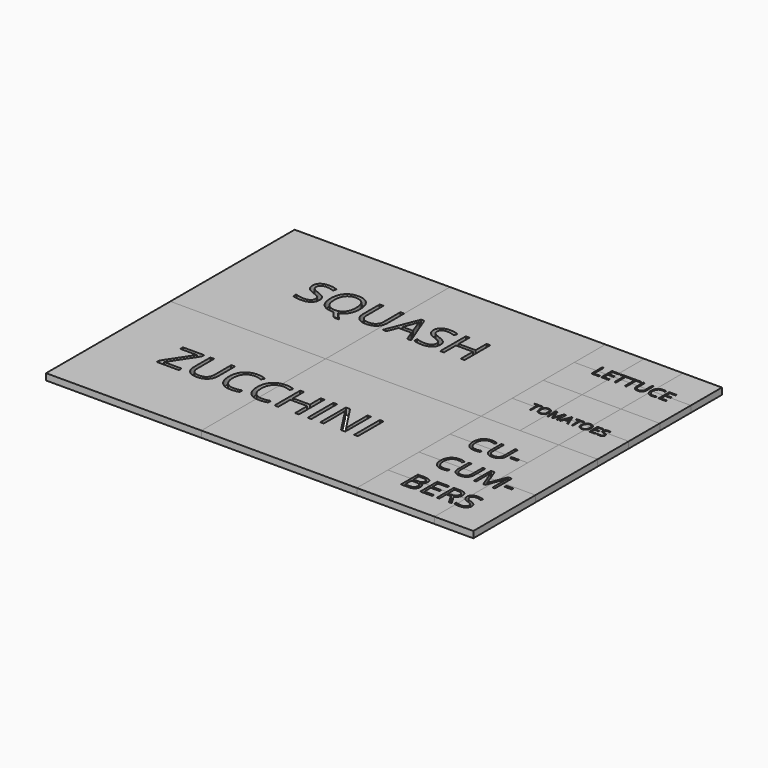
from build123d import *

# Parameters (mm, degrees)
F1_DEPTH  = 25.4
F2_DEPTH  = 25.4
F3_DEPTH  = 25.4
F0_W      = 14.634765625
F0_H      = 125.9251302083
F4_DEPTH  = 25.4
F0_W_2    = 20.5228050427
F0_H_2    = 17.0920228571
F5_DEPTH  = 25.4
F6_DEPTH  = 25.4
F7_DEPTH  = 25.4
F0_H_3    = 19.5188114286
F8_DEPTH  = 25.4
F9_DEPTH  = 25.4
F10_DEPTH = 25.4
F11_DEPTH = 25.4
F12_DEPTH = 25.4
F13_DEPTH = 25.4
F14_DEPTH = 25.4
F0_W_3    = 28.0196080781
F0_H_4    = 8.6762150177
F15_DEPTH = 25.4
F16_DEPTH = 25.4


with BuildPart() as f1:
    # F0 (on Top) → F1 (new body)
    with BuildSketch(Plane.XY):
        with BuildLine():
            Line((-44.0684282231, 324.3166356862), (-653.6684282231, 324.3166356862))
            Line((-653.6684282231, 324.3166356862), (-653.6684282231, -285.2833643138))
            Line((-653.6684282231, -285.2833643138), (-44.0684282231, -285.2833643138))
            Line((-44.0684282231, -285.2833643138), (-44.0684282231, 15.1915384778))
            add(Edge.make_bspline(
                [(-44.0684282231, 15.1915384778), (-44.9418856764, -4.1809977171), (-57.0089513169, -15.6089179317)],
                knots=[0.0723835835, 0.0723835835, 0.0723835835, 1, 1, 1], degree=2))
            add(Edge.make_bspline(
                [(-57.0089513169, -15.6089179317), (-70.0176318724, -27.92857939), (-92.7552620808, -27.92857939)],
                knots=[0, 0, 0, 1, 1, 1], degree=2))
            add(Edge.make_bspline(
                [(-92.7552620808, -27.92857939), (-115.4928922891, -27.92857939), (-127.9365771849, -15.5124552581)],
                knots=[0, 0, 0, 1, 1, 1], degree=2))
            add(Edge.make_bspline(
                [(-127.9365771849, -15.5124552581), (-140.3802620808, -3.0963311262), (-140.3802620808, 18.5939900544)],
                knots=[0, 0, 0, 1, 1, 1], degree=2))
            Line((-140.3802620808, 18.5939900544), (-140.3802620808, 99.7328789433))
            Line((-140.3802620808, 99.7328789433), (-125.7179356919, 99.7328789433))
            Line((-125.7179356919, 99.7328789433), (-125.7179356919, 17.5742417905))
            add(Edge.make_bspline(
                [(-125.7179356919, 17.5742417905), (-125.7179356919, 1.8094848461), (-117.1051969766, -6.6378892859)],
                knots=[0, 0, 0, 1, 1, 1], degree=2))
            add(Edge.make_bspline(
                [(-117.1051969766, -6.6378892859), (-108.4924582613, -15.0852634178), (-91.7906353446, -15.0852634178)],
                knots=[0, 0, 0, 1, 1, 1], degree=2))
            add(Edge.make_bspline(
                [(-91.7906353446, -15.0852634178), (-75.8605138169, -15.0852634178), (-67.2477751016, -6.59654814)],
                knots=[0, 0, 0, 1, 1, 1], degree=2))
            add(Edge.make_bspline(
                [(-67.2477751016, -6.59654814), (-58.6350363863, 1.8921671377), (-58.6350363863, 17.7396063738)],
                knots=[0, 0, 0, 1, 1, 1], degree=2))
            Line((-58.6350363863, 17.7396063738), (-58.6350363863, 99.7328789433))
            Line((-58.6350363863, 99.7328789433), (-44.0684282231, 99.7328789433))
            Line((-44.0684282231, 99.7328789433), (-44.0684282231, 324.3166356862))
        make_face()
        with BuildLine():
            add(Edge.make_bspline(
                [(-309.6584738863, 28.3229397072), (-302.2170676363, 20.2200751238), (-302.2170676363, 7.3216376238)],
                knots=[0, 0, 0, 1, 1, 1], degree=2))
            add(Edge.make_bspline(
                [(-302.2170676363, 7.3216376238), (-302.2170676363, -9.2975030012), (-314.2749018377, -18.6130411956)],
                knots=[0, 0, 0, 1, 1, 1], degree=2))
            add(Edge.make_bspline(
                [(-314.2749018377, -18.6130411956), (-326.3327360391, -27.92857939), (-347.0033089558, -27.92857939)],
                knots=[0, 0, 0, 1, 1, 1], degree=2))
            add(Edge.make_bspline(
                [(-347.0033089558, -27.92857939), (-369.3826492335, -27.92857939), (-381.4542638169, -22.1408189734)],
                knots=[0, 0, 0, 1, 1, 1], degree=2))
            Line((-381.4542638169, -22.1408189734), (-381.4542638169, -8.0297078623))
            add(Edge.make_bspline(
                [(-381.4542638169, -8.0297078623), (-373.6821284002, -11.2818780012), (-364.559515553, -13.1835707095)],
                knots=[0, 0, 0, 1, 1, 1], degree=2))
            add(Edge.make_bspline(
                [(-364.559515553, -13.1835707095), (-355.4369027058, -15.0852634178), (-346.4796544419, -15.0852634178)],
                knots=[0, 0, 0, 1, 1, 1], degree=2))
            add(Edge.make_bspline(
                [(-346.4796544419, -15.0852634178), (-331.8448888169, -15.0852634178), (-324.4310433308, -9.5317694942)],
                knots=[0, 0, 0, 1, 1, 1], degree=2))
            add(Edge.make_bspline(
                [(-324.4310433308, -9.5317694942), (-317.0171978446, -3.9782755706), (-317.0171978446, 5.9435994294)],
                knots=[0, 0, 0, 1, 1, 1], degree=2))
            add(Edge.make_bspline(
                [(-317.0171978446, 5.9435994294), (-317.0171978446, 12.4755004711), (-319.649250796, 16.6509562002)],
                knots=[0, 0, 0, 1, 1, 1], degree=2))
            add(Edge.make_bspline(
                [(-319.649250796, 16.6509562002), (-322.2813037474, 20.8264119294), (-328.4411344766, 24.3679700891)],
                knots=[0, 0, 0, 1, 1, 1], degree=2))
            add(Edge.make_bspline(
                [(-328.4411344766, 24.3679700891), (-334.6009652058, 27.9095282488), (-347.1686735391, 32.3743719988)],
                knots=[0, 0, 0, 1, 1, 1], degree=2))
            add(Edge.make_bspline(
                [(-347.1686735391, 32.3743719988), (-364.7248801363, 38.6582261655), (-372.2627490599, 47.2709648808)],
                knots=[0, 0, 0, 1, 1, 1], degree=2))
            add(Edge.make_bspline(
                [(-372.2627490599, 47.2709648808), (-379.8006179835, 55.8837035961), (-379.8006179835, 69.7467678322)],
                knots=[0, 0, 0, 1, 1, 1], degree=2))
            add(Edge.make_bspline(
                [(-379.8006179835, 69.7467678322), (-379.8006179835, 84.2988511655), (-368.8727751016, 92.9115898808)],
                knots=[0, 0, 0, 1, 1, 1], degree=2))
            add(Edge.make_bspline(
                [(-368.8727751016, 92.9115898808), (-357.9449322196, 101.5243285961), (-339.9201926363, 101.5243285961)],
                knots=[0, 0, 0, 1, 1, 1], degree=2))
            add(Edge.make_bspline(
                [(-339.9201926363, 101.5243285961), (-321.151312428, 101.5243285961), (-305.3865554835, 94.6341376238)],
                knots=[0, 0, 0, 1, 1, 1], degree=2))
            Line((-305.3865554835, 94.6341376238), (-309.9616422891, 81.9010647072))
            add(Edge.make_bspline(
                [(-309.9616422891, 81.9010647072), (-325.5610346502, 88.4329657488), (-340.2784825669, 88.4329657488)],
                knots=[0, 0, 0, 1, 1, 1], degree=2))
            add(Edge.make_bspline(
                [(-340.2784825669, 88.4329657488), (-351.909124928, 88.4329657488), (-358.4548063516, 83.444467485)],
                knots=[0, 0, 0, 1, 1, 1], degree=2))
            add(Edge.make_bspline(
                [(-358.4548063516, 83.444467485), (-365.0004877752, 78.4559692211), (-365.0004877752, 69.5814032488)],
                knots=[0, 0, 0, 1, 1, 1], degree=2))
            add(Edge.make_bspline(
                [(-365.0004877752, 69.5814032488), (-365.0004877752, 63.0495022072), (-362.5889209349, 58.8602660961)],
                knots=[0, 0, 0, 1, 1, 1], degree=2))
            add(Edge.make_bspline(
                [(-362.5889209349, 58.8602660961), (-360.1773540946, 54.671029985), (-354.4447152058, 51.184593353)],
                knots=[0, 0, 0, 1, 1, 1], degree=2))
            add(Edge.make_bspline(
                [(-354.4447152058, 51.184593353), (-348.7120763169, 47.6981567211), (-336.9160693724, 43.4813598461)],
                knots=[0, 0, 0, 1, 1, 1], degree=2))
            add(Edge.make_bspline(
                [(-336.9160693724, 43.4813598461), (-317.0998801363, 36.4258042905), (-309.6584738863, 28.3229397072)],
                knots=[0, 0, 0, 1, 1, 1], degree=2))
        make_face(mode=Mode.SUBTRACT)
        with BuildLine():
            add(Edge.make_bspline(
                [(-182.3828662474, 84.4917765127), (-167.1417638169, 67.2662990822), (-167.1417638169, 36.9494588044)],
                knots=[0, 0, 0, 1, 1, 1], degree=2))
            add(Edge.make_bspline(
                [(-167.1417638169, 36.9494588044), (-167.1417638169, 12.75110811), (-176.8707134696, -3.2754760914)],
                knots=[0, 0, 0, 1, 1, 1], degree=2))
            add(Edge.make_bspline(
                [(-176.8707134696, -3.2754760914), (-186.5996631224, -19.3020602928), (-204.3487950669, -24.9795776539)],
                knots=[0, 0, 0, 1, 1, 1], degree=2))
            Line((-204.3487950669, -24.9795776539), (-174.3902447196, -56.1783623762))
            Line((-174.3902447196, -56.1783623762), (-195.6671544419, -56.1783623762))
            Line((-195.6671544419, -56.1783623762), (-220.196234303, -27.7356540428))
            Line((-220.196234303, -27.7356540428), (-224.9366856919, -27.92857939))
            add(Edge.make_bspline(
                [(-224.9366856919, -27.92857939), (-252.7454964558, -27.92857939), (-267.8625754488, -10.9098076887)],
                knots=[0, 0, 0, 1, 1, 1], degree=2))
            add(Edge.make_bspline(
                [(-267.8625754488, -10.9098076887), (-282.9796544419, 6.1089640127), (-282.9796544419, 37.1148233877)],
                knots=[0, 0, 0, 1, 1, 1], degree=2))
            add(Edge.make_bspline(
                [(-282.9796544419, 37.1148233877), (-282.9796544419, 67.8726358877), (-267.821234303, 84.7949449155)],
                knots=[0, 0, 0, 1, 1, 1], degree=2))
            add(Edge.make_bspline(
                [(-267.821234303, 84.7949449155), (-252.6628141641, 101.7172539433), (-224.7713211085, 101.7172539433)],
                knots=[0, 0, 0, 1, 1, 1], degree=2))
            add(Edge.make_bspline(
                [(-224.7713211085, 101.7172539433), (-197.623968678, 101.7172539433), (-182.3828662474, 84.4917765127)],
                knots=[0, 0, 0, 1, 1, 1], degree=2))
        make_face(mode=Mode.SUBTRACT)
    extrude(amount=F1_DEPTH)


with BuildPart() as f1b:
    # F0 (on Top) → F1, piece 2 (new body)
    with BuildSketch(Plane.XY):
        with BuildLine():
            add(Edge.make_bspline(
                [(-256.5902230183, 75.3967244294), (-267.4905051363, 62.1675577627), (-267.4905051363, 36.9494588044)],
                knots=[0, 0, 0, 1, 1, 1], degree=2))
            add(Edge.make_bspline(
                [(-267.4905051363, 36.9494588044), (-267.4905051363, 11.3730699155), (-256.5902230183, -1.8560967512)],
                knots=[0, 0, 0, 1, 1, 1], degree=2))
            add(Edge.make_bspline(
                [(-256.5902230183, -1.8560967512), (-245.6899409002, -15.0852634178), (-224.9366856919, -15.0852634178)],
                knots=[0, 0, 0, 1, 1, 1], degree=2))
            add(Edge.make_bspline(
                [(-224.9366856919, -15.0852634178), (-204.0180659002, -15.0852634178), (-193.3382698933, -1.9112182789)],
                knots=[0, 0, 0, 1, 1, 1], degree=2))
            add(Edge.make_bspline(
                [(-193.3382698933, -1.9112182789), (-182.6584738863, 11.26282686), (-182.6584738863, 36.9494588044)],
                knots=[0, 0, 0, 1, 1, 1], degree=2))
            add(Edge.make_bspline(
                [(-182.6584738863, 36.9494588044), (-182.6584738863, 62.36048311), (-193.2969287474, 75.493187103)],
                knots=[0, 0, 0, 1, 1, 1], degree=2))
            add(Edge.make_bspline(
                [(-193.2969287474, 75.493187103), (-203.9353836085, 88.6258910961), (-224.7713211085, 88.6258910961)],
                knots=[0, 0, 0, 1, 1, 1], degree=2))
            add(Edge.make_bspline(
                [(-224.7713211085, 88.6258910961), (-245.6899409002, 88.6258910961), (-256.5902230183, 75.3967244294)],
                knots=[0, 0, 0, 1, 1, 1], degree=2))
        make_face()
    extrude(amount=F1_DEPTH)


with BuildPart() as f2:
    # F0 (on Top) → F2 (new body)
    with BuildSketch(Plane.XY):
        with BuildLine():
            Line((7.510796947, 27.0275838044), (48.2456059748, 27.0275838044))
            Line((48.2456059748, 27.0275838044), (33.5832795859, 66.0536254711))
            add(Edge.make_bspline(
                [(33.5832795859, 66.0536254711), (30.7445209054, 73.4674709572), (27.7403976415, 84.2161688738)],
                knots=[0, 0, 0, 1, 1, 1], degree=2))
            add(Edge.make_bspline(
                [(27.7403976415, 84.2161688738), (25.8387049331, 75.9479397072), (22.3109271554, 66.0536254711)],
                knots=[0, 0, 0, 1, 1, 1], degree=2))
            Line((22.3109271554, 66.0536254711), (7.510796947, 27.0275838044))
        make_face()
    extrude(amount=F2_DEPTH)


with BuildPart() as f2b:
    # F0 (on Top) → F2, piece 2 (new body)
    with BuildSketch(Plane.XY):
        with BuildLine():
            Line((565.5315717769, 324.3166356862), (-44.0684282231, 324.3166356862))
            Line((-44.0684282231, 324.3166356862), (-44.0684282231, 99.7328789433))
            Line((-44.0684282231, 99.7328789433), (-44.0002707613, 99.7328789433))
            Line((-44.0002707613, 99.7328789433), (-44.0002707613, 18.2632608877))
            add(Edge.make_bspline(
                [(-44.0002707613, 18.2632608877), (-44.0002707613, 16.7032124479), (-44.0684282231, 15.1915384778)],
                knots=[0, 0, 0, 0.0723835835, 0.0723835835, 0.0723835835], degree=2))
            Line((-44.0684282231, 15.1915384778), (-44.0684282231, -285.2833643138))
            Line((-44.0684282231, -285.2833643138), (565.5315717769, -285.2833643138))
            Line((565.5315717769, -285.2833643138), (565.5315717769, -132.8833643138))
            Line((565.5315717769, -132.8833643138), (565.5315717769, 19.5166356861))
            Line((565.5315717769, 19.5166356861), (565.5315717769, 171.9166356862))
            Line((565.5315717769, 171.9166356862), (565.5315717769, 324.3166356862))
        make_face()
        Polygon((83.6336268081, -26.192251265), (68.4752066692, -26.192251265), (52.7931320165, 13.8535386655), (2.3293733359, 13.8535386655), (-13.1597759696, -26.192251265), (-27.9874669419, -26.192251265), (21.7872726415, 100.2565334572), (34.1069340998, 100.2565334572), align=None, mode=Mode.SUBTRACT)
        with BuildLine():
            add(Edge.make_bspline(
                [(164.5520295859, 28.3229397072), (171.9934358359, 20.2200751238), (171.9934358359, 7.3216376238)],
                knots=[0, 0, 0, 1, 1, 1], degree=2))
            add(Edge.make_bspline(
                [(171.9934358359, 7.3216376238), (171.9934358359, -9.2975030012), (159.9356016345, -18.6130411956)],
                knots=[0, 0, 0, 1, 1, 1], degree=2))
            add(Edge.make_bspline(
                [(159.9356016345, -18.6130411956), (147.8777674331, -27.92857939), (127.2071945165, -27.92857939)],
                knots=[0, 0, 0, 1, 1, 1], degree=2))
            add(Edge.make_bspline(
                [(127.2071945165, -27.92857939), (104.8278542387, -27.92857939), (92.7562396554, -22.1408189734)],
                knots=[0, 0, 0, 1, 1, 1], degree=2))
            Line((92.7562396554, -22.1408189734), (92.7562396554, -8.0297078623))
            add(Edge.make_bspline(
                [(92.7562396554, -8.0297078623), (100.528375072, -11.2818780012), (109.6509879192, -13.1835707095)],
                knots=[0, 0, 0, 1, 1, 1], degree=2))
            add(Edge.make_bspline(
                [(109.6509879192, -13.1835707095), (118.7736007665, -15.0852634178), (127.7308490304, -15.0852634178)],
                knots=[0, 0, 0, 1, 1, 1], degree=2))
            add(Edge.make_bspline(
                [(127.7308490304, -15.0852634178), (142.3656146554, -15.0852634178), (149.7794601415, -9.5317694942)],
                knots=[0, 0, 0, 1, 1, 1], degree=2))
            add(Edge.make_bspline(
                [(149.7794601415, -9.5317694942), (157.1933056276, -3.9782755706), (157.1933056276, 5.9435994294)],
                knots=[0, 0, 0, 1, 1, 1], degree=2))
            add(Edge.make_bspline(
                [(157.1933056276, 5.9435994294), (157.1933056276, 12.4755004711), (154.5612526762, 16.6509562002)],
                knots=[0, 0, 0, 1, 1, 1], degree=2))
            add(Edge.make_bspline(
                [(154.5612526762, 16.6509562002), (151.9291997248, 20.8264119294), (145.7693689956, 24.3679700891)],
                knots=[0, 0, 0, 1, 1, 1], degree=2))
            add(Edge.make_bspline(
                [(145.7693689956, 24.3679700891), (139.6095382665, 27.9095282488), (127.0418299331, 32.3743719988)],
                knots=[0, 0, 0, 1, 1, 1], degree=2))
            add(Edge.make_bspline(
                [(127.0418299331, 32.3743719988), (109.4856233359, 38.6582261655), (101.9477544123, 47.2709648808)],
                knots=[0, 0, 0, 1, 1, 1], degree=2))
            add(Edge.make_bspline(
                [(101.9477544123, 47.2709648808), (94.4098854887, 55.8837035961), (94.4098854887, 69.7467678322)],
                knots=[0, 0, 0, 1, 1, 1], degree=2))
            add(Edge.make_bspline(
                [(94.4098854887, 69.7467678322), (94.4098854887, 84.2988511655), (105.3377283706, 92.9115898808)],
                knots=[0, 0, 0, 1, 1, 1], degree=2))
            add(Edge.make_bspline(
                [(105.3377283706, 92.9115898808), (116.2655712526, 101.5243285961), (134.2903108359, 101.5243285961)],
                knots=[0, 0, 0, 1, 1, 1], degree=2))
            add(Edge.make_bspline(
                [(134.2903108359, 101.5243285961), (153.0591910442, 101.5243285961), (168.8239479887, 94.6341376238)],
                knots=[0, 0, 0, 1, 1, 1], degree=2))
            Line((168.8239479887, 94.6341376238), (164.2488611831, 81.9010647072))
            add(Edge.make_bspline(
                [(164.2488611831, 81.9010647072), (148.649468822, 88.4329657488), (133.9320209054, 88.4329657488)],
                knots=[0, 0, 0, 1, 1, 1], degree=2))
            add(Edge.make_bspline(
                [(133.9320209054, 88.4329657488), (122.3013785442, 88.4329657488), (115.7556971206, 83.444467485)],
                knots=[0, 0, 0, 1, 1, 1], degree=2))
            add(Edge.make_bspline(
                [(115.7556971206, 83.444467485), (109.210015697, 78.4559692211), (109.210015697, 69.5814032488)],
                knots=[0, 0, 0, 1, 1, 1], degree=2))
            add(Edge.make_bspline(
                [(109.210015697, 69.5814032488), (109.210015697, 63.0495022072), (111.6215825373, 58.8602660961)],
                knots=[0, 0, 0, 1, 1, 1], degree=2))
            add(Edge.make_bspline(
                [(111.6215825373, 58.8602660961), (114.0331493776, 54.671029985), (119.7657882665, 51.184593353)],
                knots=[0, 0, 0, 1, 1, 1], degree=2))
            add(Edge.make_bspline(
                [(119.7657882665, 51.184593353), (125.4984271554, 47.6981567211), (137.2944340998, 43.4813598461)],
                knots=[0, 0, 0, 1, 1, 1], degree=2))
            add(Edge.make_bspline(
                [(137.2944340998, 43.4813598461), (157.1106233359, 36.4258042905), (164.5520295859, 28.3229397072)],
                knots=[0, 0, 0, 1, 1, 1], degree=2))
        make_face(mode=Mode.SUBTRACT)
        Polygon((293.3710400026, 99.7328789433), (293.3710400026, -26.192251265), (278.7362743776, -26.192251265), (278.7362743776, 33.0633910961), (212.397515697, 33.0633910961), (212.397515697, -26.192251265), (197.762750072, -26.192251265), (197.762750072, 99.7328789433), (212.397515697, 99.7328789433), (212.397515697, 46.1547539433), (278.7362743776, 46.1547539433), (278.7362743776, 99.7328789433), align=None, mode=Mode.SUBTRACT)
    extrude(amount=F2_DEPTH)


with BuildPart() as f3:
    # F0 (on Top) → F3 (new body)
    with BuildSketch(Plane.XY):
        with BuildLine():
            Line((-44.0684282231, -612.1363602298), (-44.0684282231, -511.9295382423))
            add(Edge.make_bspline(
                [(-44.0684282231, -511.9295382423), (-55.6579949116, -515.0582749205), (-63.5136684446, -524.0941012435)],
                knots=[0.3462590544, 0.3462590544, 0.3462590544, 1, 1, 1], degree=2))
            add(Edge.make_bspline(
                [(-63.5136684446, -524.0941012435), (-75.5301615002, -537.9158243338), (-75.5301615002, -561.9488104449)],
                knots=[0, 0, 0, 1, 1, 1], degree=2))
            add(Edge.make_bspline(
                [(-75.5301615002, -561.9488104449), (-75.5301615002, -586.6432548894), (-63.9408602849, -600.134248813)],
                knots=[0, 0, 0, 1, 1, 1], degree=2))
            add(Edge.make_bspline(
                [(-63.9408602849, -600.134248813), (-56.2016012803, -609.1434456804), (-44.0684282231, -612.1363602298)],
                knots=[0, 0, 0, 0.6677934123, 0.6677934123, 0.6677934123], degree=2))
        make_face()
    extrude(amount=F3_DEPTH)


with BuildPart() as f3b:
    # F0 (on Top) → F3, piece 2 (new body)
    with BuildSketch(Plane.XY):
        with BuildLine():
            Line((-44.0684282231, -285.2833643138), (-653.6684282231, -285.2833643138))
            Line((-653.6684282231, -285.2833643138), (-653.6684282231, -894.8833643138))
            Line((-653.6684282231, -894.8833643138), (-44.0684282231, -894.8833643138))
            Line((-44.0684282231, -894.8833643138), (-44.0684282231, -625.9158614052))
            add(Edge.make_bspline(
                [(-44.0684282231, -625.9158614052), (-64.0670592157, -623.1508966172), (-76.067596396, -609.7391750283)],
                knots=[0.206160318, 0.206160318, 0.206160318, 1, 1, 1], degree=2))
            add(Edge.make_bspline(
                [(-76.067596396, -609.7391750283), (-91.1846753891, -592.8444267644), (-91.1846753891, -561.7558850977)],
                knots=[0, 0, 0, 1, 1, 1], degree=2))
            add(Edge.make_bspline(
                [(-91.1846753891, -561.7558850977), (-91.1846753891, -542.2979857922), (-83.9086337224, -527.6632201672)],
                knots=[0, 0, 0, 1, 1, 1], degree=2))
            add(Edge.make_bspline(
                [(-83.9086337224, -527.6632201672), (-76.6325920557, -513.0284545422), (-62.8935512571, -505.1047349241)],
                knots=[0, 0, 0, 1, 1, 1], degree=2))
            add(Edge.make_bspline(
                [(-62.8935512571, -505.1047349241), (-54.4086460934, -500.2112339521), (-44.0684282231, -498.3398429129)],
                knots=[0, 0, 0, 0.6175762404, 0.6175762404, 0.6175762404], degree=2))
            Line((-44.0684282231, -498.3398429129), (-44.0684282231, -285.2833643138))
        make_face()
        Polygon((-348.7124531669, -611.6408677366), (-348.7124531669, -624.8975951672), (-435.2808125419, -624.8975951672), (-435.2808125419, -613.4323173894), (-368.4459601113, -512.1465100977), (-433.2137552502, -512.1465100977), (-433.2137552502, -498.9724649588), (-350.6141458752, -498.9724649588), (-350.6141458752, -510.4377427366), (-417.4489983057, -611.6408677366), align=None, mode=Mode.SUBTRACT)
        with BuildLine():
            Line((-243.8988680974, -498.9724649588), (-229.2641024724, -498.9724649588))
            Line((-229.2641024724, -498.9724649588), (-229.2641024724, -580.4420830144))
            add(Edge.make_bspline(
                [(-229.2641024724, -580.4420830144), (-229.2641024724, -601.9946003755), (-242.272783028, -614.3142618338)],
                knots=[0, 0, 0, 1, 1, 1], degree=2))
            add(Edge.make_bspline(
                [(-242.272783028, -614.3142618338), (-255.2814635835, -626.6339232922), (-278.0190937919, -626.6339232922)],
                knots=[0, 0, 0, 1, 1, 1], degree=2))
            add(Edge.make_bspline(
                [(-278.0190937919, -626.6339232922), (-300.7567240002, -626.6339232922), (-313.200408896, -614.2177991602)],
                knots=[0, 0, 0, 1, 1, 1], degree=2))
            add(Edge.make_bspline(
                [(-313.200408896, -614.2177991602), (-325.6440937919, -601.8016750283), (-325.6440937919, -580.1113538477)],
                knots=[0, 0, 0, 1, 1, 1], degree=2))
            Line((-325.6440937919, -580.1113538477), (-325.6440937919, -498.9724649588))
            Line((-325.6440937919, -498.9724649588), (-310.981767403, -498.9724649588))
            Line((-310.981767403, -498.9724649588), (-310.981767403, -581.1311021116))
            add(Edge.make_bspline(
                [(-310.981767403, -581.1311021116), (-310.981767403, -596.895859056), (-302.3690286877, -605.343233188)],
                knots=[0, 0, 0, 1, 1, 1], degree=2))
            add(Edge.make_bspline(
                [(-302.3690286877, -605.343233188), (-293.7562899724, -613.7906073199), (-277.0544670557, -613.7906073199)],
                knots=[0, 0, 0, 1, 1, 1], degree=2))
            add(Edge.make_bspline(
                [(-277.0544670557, -613.7906073199), (-261.124345528, -613.7906073199), (-252.5116068127, -605.3018920422)],
                knots=[0, 0, 0, 1, 1, 1], degree=2))
            add(Edge.make_bspline(
                [(-252.5116068127, -605.3018920422), (-243.8988680974, -596.8131767644), (-243.8988680974, -580.9657375283)],
                knots=[0, 0, 0, 1, 1, 1], degree=2))
            Line((-243.8988680974, -580.9657375283), (-243.8988680974, -498.9724649588))
        make_face(mode=Mode.SUBTRACT)
        with BuildLine():
            add(Edge.make_bspline(
                [(-113.4262118474, -516.9696437783), (-127.7302483057, -510.2723781533), (-142.0342847641, -510.2723781533)],
                knots=[0, 0, 0, 1, 1, 1], degree=2))
            add(Edge.make_bspline(
                [(-142.0342847641, -510.2723781533), (-162.7875399724, -510.2723781533), (-174.804033028, -524.0941012435)],
                knots=[0, 0, 0, 1, 1, 1], degree=2))
            add(Edge.make_bspline(
                [(-174.804033028, -524.0941012435), (-186.8205260835, -537.9158243338), (-186.8205260835, -561.9488104449)],
                knots=[0, 0, 0, 1, 1, 1], degree=2))
            add(Edge.make_bspline(
                [(-186.8205260835, -561.9488104449), (-186.8205260835, -586.6432548894), (-175.2312248682, -600.134248813)],
                knots=[0, 0, 0, 1, 1, 1], degree=2))
            add(Edge.make_bspline(
                [(-175.2312248682, -600.134248813), (-163.641923653, -613.6252427366), (-142.1996493474, -613.6252427366)],
                knots=[0, 0, 0, 1, 1, 1], degree=2))
            add(Edge.make_bspline(
                [(-142.1996493474, -613.6252427366), (-129.0256042085, -613.6252427366), (-112.1308559446, -608.8847913477)],
                knots=[0, 0, 0, 1, 1, 1], degree=2))
            Line((-112.1308559446, -608.8847913477), (-112.1308559446, -621.700546556))
            add(Edge.make_bspline(
                [(-112.1308559446, -621.700546556), (-125.2222187919, -626.6339232922), (-144.4320712224, -626.6339232922)],
                knots=[0, 0, 0, 1, 1, 1], degree=2))
            add(Edge.make_bspline(
                [(-144.4320712224, -626.6339232922), (-172.2408819863, -626.6339232922), (-187.3579609794, -609.7391750283)],
                knots=[0, 0, 0, 1, 1, 1], degree=2))
            add(Edge.make_bspline(
                [(-187.3579609794, -609.7391750283), (-202.4750399724, -592.8444267644), (-202.4750399724, -561.7558850977)],
                knots=[0, 0, 0, 1, 1, 1], degree=2))
            add(Edge.make_bspline(
                [(-202.4750399724, -561.7558850977), (-202.4750399724, -542.2979857922), (-195.1989983057, -527.6632201672)],
                knots=[0, 0, 0, 1, 1, 1], degree=2))
            add(Edge.make_bspline(
                [(-195.1989983057, -527.6632201672), (-187.9229566391, -513.0284545422), (-174.1839158405, -505.1047349241)],
                knots=[0, 0, 0, 1, 1, 1], degree=2))
            add(Edge.make_bspline(
                [(-174.1839158405, -505.1047349241), (-160.4448750419, -497.181015306), (-141.8413594169, -497.181015306)],
                knots=[0, 0, 0, 1, 1, 1], degree=2))
            add(Edge.make_bspline(
                [(-141.8413594169, -497.181015306), (-122.0527309446, -497.181015306), (-107.2250399724, -504.4019354449)],
                knots=[0, 0, 0, 1, 1, 1], degree=2))
            Line((-107.2250399724, -504.4019354449), (-113.4262118474, -516.9696437783))
        make_face(mode=Mode.SUBTRACT)
    extrude(amount=F3_DEPTH)


with BuildPart() as f4:
    # F0 (on Top) → F4 (new body)
    with BuildSketch(Plane.XY):
        with BuildLine():
            Line((565.5315717769, -285.2833643138), (-44.0684282231, -285.2833643138))
            Line((-44.0684282231, -285.2833643138), (-44.0684282231, -498.3398429129))
            add(Edge.make_bspline(
                [(-44.0684282231, -498.3398429129), (-37.6654212198, -497.181015306), (-30.5509948335, -497.181015306)],
                knots=[0.6175762404, 0.6175762404, 0.6175762404, 1, 1, 1], degree=2))
            add(Edge.make_bspline(
                [(-30.5509948335, -497.181015306), (-10.7623663613, -497.181015306), (4.0653246109, -504.4019354449)],
                knots=[0, 0, 0, 1, 1, 1], degree=2))
            Line((4.0653246109, -504.4019354449), (-2.1358472641, -516.9696437783))
            add(Edge.make_bspline(
                [(-2.1358472641, -516.9696437783), (-16.4398837224, -510.2723781533), (-30.7439201807, -510.2723781533)],
                knots=[0, 0, 0, 1, 1, 1], degree=2))
            add(Edge.make_bspline(
                [(-30.7439201807, -510.2723781533), (-37.9299227047, -510.2723781533), (-44.0684282231, -511.9295382423)],
                knots=[0, 0, 0, 0.3462590544, 0.3462590544, 0.3462590544], degree=2))
            Line((-44.0684282231, -511.9295382423), (-44.0684282231, -612.1363602298))
            add(Edge.make_bspline(
                [(-44.0684282231, -612.1363602298), (-38.0325495439, -613.6252427366), (-30.9092847641, -613.6252427366)],
                knots=[0.6677934123, 0.6677934123, 0.6677934123, 1, 1, 1], degree=2))
            add(Edge.make_bspline(
                [(-30.9092847641, -613.6252427366), (-17.7352396252, -613.6252427366), (-0.8404913613, -608.8847913477)],
                knots=[0, 0, 0, 1, 1, 1], degree=2))
            Line((-0.8404913613, -608.8847913477), (-0.8404913613, -621.700546556))
            add(Edge.make_bspline(
                [(-0.8404913613, -621.700546556), (-13.9318542085, -626.6339232922), (-33.1417066391, -626.6339232922)],
                knots=[0, 0, 0, 1, 1, 1], degree=2))
            add(Edge.make_bspline(
                [(-33.1417066391, -626.6339232922), (-38.8747799099, -626.6339232922), (-44.0684282231, -625.9158614052)],
                knots=[0, 0, 0, 0.206160318, 0.206160318, 0.206160318], degree=2))
            Line((-44.0684282231, -625.9158614052), (-44.0684282231, -894.8833643138))
            Line((-44.0684282231, -894.8833643138), (565.5315717769, -894.8833643138))
            Line((565.5315717769, -894.8833643138), (565.5315717769, -742.4833643138))
            Line((565.5315717769, -742.4833643138), (565.5315717769, -590.0833643138))
            Line((565.5315717769, -590.0833643138), (565.5315717769, -437.6833643138))
            Line((565.5315717769, -437.6833643138), (565.5315717769, -285.2833643138))
        make_face()
        Polygon((122.2458801665, -498.9724649588), (122.2458801665, -624.8975951672), (107.6111145415, -624.8975951672), (107.6111145415, -565.641952806), (41.2723558609, -565.641952806), (41.2723558609, -624.8975951672), (26.6375902359, -624.8975951672), (26.6375902359, -498.9724649588), (41.2723558609, -498.9724649588), (41.2723558609, -552.5505899588), (107.6111145415, -552.5505899588), (107.6111145415, -498.9724649588), align=None, mode=Mode.SUBTRACT)
        with Locations((164.0969001318, -561.935030063)):
            Rectangle(F0_W, F0_H, mode=Mode.SUBTRACT)
        with BuildLine():
            Line((304.3122864165, -498.9724649588), (304.3122864165, -624.8975951672))
            Line((304.3122864165, -624.8975951672), (287.6104634998, -624.8975951672))
            Line((287.6104634998, -624.8975951672), (218.7912360693, -519.2296264172))
            Line((218.7912360693, -519.2296264172), (218.102216972, -519.2296264172))
            add(Edge.make_bspline(
                [(218.102216972, -519.2296264172), (219.4802551665, -537.8331420422), (219.4802551665, -553.3222913477)],
                knots=[0, 0, 0, 1, 1, 1], degree=2))
            Line((219.4802551665, -553.3222913477), (219.4802551665, -624.8975951672))
            Line((219.4802551665, -624.8975951672), (205.947920097, -624.8975951672))
            Line((205.947920097, -624.8975951672), (205.947920097, -498.9724649588))
            Line((205.947920097, -498.9724649588), (222.4843784304, -498.9724649588))
            Line((222.4843784304, -498.9724649588), (291.1382412776, -604.2270222505))
            Line((291.1382412776, -604.2270222505), (291.8272603748, -604.2270222505))
            add(Edge.make_bspline(
                [(291.8272603748, -604.2270222505), (291.6618957915, -601.9119180838), (291.0555589859, -589.2890882227)],
                knots=[0, 0, 0, 1, 1, 1], degree=2))
            add(Edge.make_bspline(
                [(291.0555589859, -589.2890882227), (290.4492221804, -576.6662583616), (290.6145867637, -571.2367878755)],
                knots=[0, 0, 0, 1, 1, 1], degree=2))
            Line((290.6145867637, -571.2367878755), (290.6145867637, -498.9724649588))
            Line((290.6145867637, -498.9724649588), (304.3122864165, -498.9724649588))
        make_face(mode=Mode.SUBTRACT)
        with Locations((346.2459886734, -561.935030063)):
            Rectangle(F0_W, F0_H, mode=Mode.SUBTRACT)
    extrude(amount=F4_DEPTH)


with BuildPart() as f5:
    # F0 (on Top) → F5 (new body)
    with BuildSketch(Plane.XY):
        with Locations((707.6701692555, 185.5426471147)):
            Rectangle(F0_W_2, F0_H_2)
    extrude(amount=F5_DEPTH)


with BuildPart() as f5b:
    # F0 (on Top) → F5, piece 2 (new body)
    with BuildSketch(Plane.XY):
        Polygon((717.9315717769, 324.3166356862), (565.5315717769, 324.3166356862), (565.5315717769, 171.9166356862), (652.6699324484, 171.9166356862), (652.6699324484, 199.569252829), (658.8356010199, 199.569252829), (658.8356010199, 171.9166356862), (691.2430981627, 171.9166356862), (691.2430981627, 199.569252829), (717.9315717769, 199.569252829), align=None)
    extrude(amount=F5_DEPTH)


with BuildPart() as f6:
    # F0 (on Top) → F6 (new body)
    with BuildSketch(Plane.XY):
        with BuildLine():
            Line((870.3315717769, 324.3166356862), (717.9315717769, 324.3166356862))
            Line((717.9315717769, 324.3166356862), (717.9315717769, 199.569252829))
            Line((717.9315717769, 199.569252829), (720.8174067341, 199.569252829))
            Line((720.8174067341, 199.569252829), (720.8174067341, 194.0886585433))
            Line((720.8174067341, 194.0886585433), (717.9315717769, 194.0886585433))
            Line((717.9315717769, 194.0886585433), (717.9315717769, 176.9966356861))
            Line((717.9315717769, 176.9966356861), (719.4008124484, 176.9966356861))
            Line((719.4008124484, 176.9966356861), (719.4008124484, 171.9166356862))
            Line((719.4008124484, 171.9166356862), (742.7281724484, 171.9166356862))
            Line((742.7281724484, 171.9166356862), (742.7281724484, 194.0886585433))
            Line((742.7281724484, 194.0886585433), (725.9264353056, 194.0886585433))
            Line((725.9264353056, 194.0886585433), (725.9264353056, 199.569252829))
            Line((725.9264353056, 199.569252829), (765.6955781627, 199.569252829))
            Line((765.6955781627, 199.569252829), (765.6955781627, 194.0886585433))
            Line((765.6955781627, 194.0886585433), (748.8938410199, 194.0886585433))
            Line((748.8938410199, 194.0886585433), (748.8938410199, 171.9166356862))
            Line((748.8938410199, 171.9166356862), (783.8442410199, 171.9166356862))
            Line((783.8442410199, 171.9166356862), (783.8442410199, 194.0886585433))
            Line((783.8442410199, 194.0886585433), (767.042503877, 194.0886585433))
            Line((767.042503877, 194.0886585433), (767.042503877, 199.569252829))
            Line((767.042503877, 199.569252829), (806.8116467341, 199.569252829))
            Line((806.8116467341, 199.569252829), (806.8116467341, 194.0886585433))
            Line((806.8116467341, 194.0886585433), (790.0099095913, 194.0886585433))
            Line((790.0099095913, 194.0886585433), (790.0099095913, 171.9166356862))
            Line((790.0099095913, 171.9166356862), (814.2545724484, 171.9166356862))
            Line((814.2545724484, 171.9166356862), (814.2545724484, 199.569252829))
            Line((814.2545724484, 199.569252829), (820.4318524484, 199.569252829))
            Line((820.4318524484, 199.569252829), (820.4318524484, 171.9166356862))
            Line((820.4318524484, 171.9166356862), (848.6940695913, 171.9166356862))
            Line((848.6940695913, 171.9166356862), (848.6940695913, 199.569252829))
            Line((848.6940695913, 199.569252829), (854.8597381627, 199.569252829))
            Line((854.8597381627, 199.569252829), (854.8597381627, 171.9166356862))
            Line((854.8597381627, 171.9166356862), (866.1597400245, 171.9166356862))
            add(Edge.make_bspline(
                [(866.1597400245, 171.9166356862), (866.1460467341, 172.5110986329), (866.1460467341, 173.1184185433)],
                knots=[0.9536315301, 0.9536315301, 0.9536315301, 1, 1, 1], degree=2))
            add(Edge.make_bspline(
                [(866.1460467341, 173.1184185433), (866.1460467341, 181.3160871147), (869.211463877, 187.4817556861)],
                knots=[0, 0, 0, 1, 1, 1], degree=2))
            add(Edge.make_bspline(
                [(869.211463877, 187.4817556861), (869.7322263225, 188.5291983321), (870.3315717769, 189.4950419902)],
                knots=[0, 0, 0, 0.1698830603, 0.1698830603, 0.1698830603], degree=2))
            Line((870.3315717769, 189.4950419902), (870.3315717769, 324.3166356862))
        make_face()
    extrude(amount=F6_DEPTH)


with BuildPart() as f7:
    # F0 (on Top) → F7 (new body)
    with BuildSketch(Plane.XY):
        with BuildLine():
            Line((1022.7315717769, 324.3166356862), (870.3315717769, 324.3166356862))
            Line((870.3315717769, 324.3166356862), (870.3315717769, 189.4950419902))
            add(Edge.make_bspline(
                [(870.3315717769, 189.4950419902), (873.2602146527, 194.214542451), (878.0651781627, 196.9857099718)],
                knots=[0.1698830603, 0.1698830603, 0.1698830603, 1, 1, 1], degree=2))
            add(Edge.make_bspline(
                [(878.0651781627, 196.9857099718), (883.8534753056, 200.3239956861), (891.6911895913, 200.3239956861)],
                knots=[0, 0, 0, 1, 1, 1], degree=2))
            add(Edge.make_bspline(
                [(891.6911895913, 200.3239956861), (900.0281953056, 200.3239956861), (906.275143877, 197.2818014004)],
                knots=[0, 0, 0, 1, 1, 1], degree=2))
            Line((906.275143877, 197.2818014004), (903.6625724484, 191.9869899718))
            add(Edge.make_bspline(
                [(903.6625724484, 191.9869899718), (897.6362410199, 194.8085671147), (891.6099095913, 194.8085671147)],
                knots=[0, 0, 0, 1, 1, 1], degree=2))
            add(Edge.make_bspline(
                [(891.6099095913, 194.8085671147), (882.866503877, 194.8085671147), (877.8039210199, 188.9854356861)],
                knots=[0, 0, 0, 1, 1, 1], degree=2))
            add(Edge.make_bspline(
                [(877.8039210199, 188.9854356861), (872.7413381627, 183.1623042576), (872.7413381627, 173.0371385433)],
                knots=[0, 0, 0, 1, 1, 1], degree=2))
            add(Edge.make_bspline(
                [(872.7413381627, 173.0371385433), (872.7413381627, 172.4698708663), (872.7558539435, 171.9166356862)],
                knots=[0, 0, 0, 0.0545248367, 0.0545248367, 0.0545248367], degree=2))
            Line((872.7558539435, 171.9166356862), (915.784903877, 171.9166356862))
            Line((915.784903877, 171.9166356862), (915.784903877, 199.569252829))
            Line((915.784903877, 199.569252829), (945.3592124484, 199.569252829))
            Line((945.3592124484, 199.569252829), (945.3592124484, 194.0886585433))
            Line((945.3592124484, 194.0886585433), (921.9505724484, 194.0886585433))
            Line((921.9505724484, 194.0886585433), (921.9505724484, 176.9966356861))
            Line((921.9505724484, 176.9966356861), (943.9426181627, 176.9966356861))
            Line((943.9426181627, 176.9966356861), (943.9426181627, 171.9166356862))
            Line((943.9426181627, 171.9166356862), (1022.7315717769, 171.9166356862))
            Line((1022.7315717769, 171.9166356862), (1022.7315717769, 324.3166356862))
        make_face()
    extrude(amount=F7_DEPTH)


with BuildPart() as f8:
    # F0 (on Top) → F8 (new body)
    with BuildSketch(Plane.XY):
        with Locations((707.6701692555, 161.7914699718)):
            Rectangle(F0_W_2, F0_H_3)
    extrude(amount=F8_DEPTH)


with BuildPart() as f8b:
    # F0 (on Top) → F8, piece 2 (new body)
    with BuildSketch(Plane.XY):
        Polygon((652.6699324484, 171.9166356862), (565.5315717769, 171.9166356862), (565.5315717769, 19.5166356861), (717.9315717769, 19.5166356861), (717.9315717769, 146.5166356861), (691.2430981627, 146.5166356861), (691.2430981627, 171.9166356862), (658.8356010199, 171.9166356862), (658.8356010199, 152.101732829), (682.2442410199, 152.101732829), (682.2442410199, 146.5166356861), (652.6699324484, 146.5166356861), align=None)
    extrude(amount=F8_DEPTH)


with BuildPart() as f9:
    # F0 (on Top) → F9 (new body)
    with BuildSketch(Plane.XY):
        with BuildLine():
            Line((848.6940695913, 165.025252829), (848.6940695913, 171.9166356862))
            Line((848.6940695913, 171.9166356862), (820.4318524484, 171.9166356862))
            Line((820.4318524484, 171.9166356862), (820.4318524484, 164.9555842576))
            add(Edge.make_bspline(
                [(820.4318524484, 164.9555842576), (820.4318524484, 158.3138471147), (824.060423877, 154.7549442576)],
                knots=[0, 0, 0, 1, 1, 1], degree=2))
            add(Edge.make_bspline(
                [(824.060423877, 154.7549442576), (827.6889953056, 151.1960414004), (834.7255210199, 151.1960414004)],
                knots=[0, 0, 0, 1, 1, 1], degree=2))
            add(Edge.make_bspline(
                [(834.7255210199, 151.1960414004), (841.4369267341, 151.1960414004), (845.0654981627, 154.7723614004)],
                knots=[0, 0, 0, 1, 1, 1], degree=2))
            add(Edge.make_bspline(
                [(845.0654981627, 154.7723614004), (848.6940695913, 158.3486814004), (848.6940695913, 165.025252829)],
                knots=[0, 0, 0, 1, 1, 1], degree=2))
        make_face()
    extrude(amount=F9_DEPTH)


with BuildPart() as f9b:
    # F0 (on Top) → F9, piece 2 (new body)
    with BuildSketch(Plane.XY):
        with BuildLine():
            Line((717.9315717769, 146.5166356861), (717.9315717769, 19.5166356861))
            Line((717.9315717769, 19.5166356861), (870.3315717769, 19.5166356861))
            Line((870.3315717769, 19.5166356861), (870.3315717769, 155.8125121903))
            add(Edge.make_bspline(
                [(870.3315717769, 155.8125121903), (866.3854493439, 162.1179807264), (866.1597400245, 171.9166356862)],
                knots=[0.189330509, 0.189330509, 0.189330509, 0.9536315301, 0.9536315301, 0.9536315301], degree=2))
            Line((866.1597400245, 171.9166356862), (854.8597381627, 171.9166356862))
            Line((854.8597381627, 171.9166356862), (854.8597381627, 165.2458699718))
            add(Edge.make_bspline(
                [(854.8597381627, 165.2458699718), (854.8597381627, 156.165732829), (849.379143877, 150.9754242576)],
                knots=[0, 0, 0, 1, 1, 1], degree=2))
            add(Edge.make_bspline(
                [(849.379143877, 150.9754242576), (843.8985495913, 145.7851156861), (834.3191210199, 145.7851156861)],
                knots=[0, 0, 0, 1, 1, 1], degree=2))
            add(Edge.make_bspline(
                [(834.3191210199, 145.7851156861), (824.7396924484, 145.7851156861), (819.4971324484, 151.0160642576)],
                knots=[0, 0, 0, 1, 1, 1], degree=2))
            add(Edge.make_bspline(
                [(819.4971324484, 151.0160642576), (814.2545724484, 156.247012829), (814.2545724484, 165.3852071147)],
                knots=[0, 0, 0, 1, 1, 1], degree=2))
            Line((814.2545724484, 165.3852071147), (814.2545724484, 171.9166356862))
            Line((814.2545724484, 171.9166356862), (790.0099095913, 171.9166356862))
            Line((790.0099095913, 171.9166356862), (790.0099095913, 146.5166356861))
            Line((790.0099095913, 146.5166356861), (783.8442410199, 146.5166356861))
            Line((783.8442410199, 146.5166356861), (783.8442410199, 171.9166356862))
            Line((783.8442410199, 171.9166356862), (748.8938410199, 171.9166356862))
            Line((748.8938410199, 171.9166356862), (748.8938410199, 146.5166356861))
            Line((748.8938410199, 146.5166356861), (742.7281724484, 146.5166356861))
            Line((742.7281724484, 146.5166356861), (742.7281724484, 171.9166356862))
            Line((742.7281724484, 171.9166356862), (719.4008124484, 171.9166356862))
            Line((719.4008124484, 171.9166356862), (719.4008124484, 171.5508756861))
            Line((719.4008124484, 171.5508756861), (717.9315717769, 171.5508756861))
            Line((717.9315717769, 171.5508756861), (717.9315717769, 152.0320642576))
            Line((717.9315717769, 152.0320642576), (720.8174067341, 152.0320642576))
            Line((720.8174067341, 152.0320642576), (720.8174067341, 146.5166356861))
            Line((720.8174067341, 146.5166356861), (717.9315717769, 146.5166356861))
        make_face()
    extrude(amount=F9_DEPTH)


with BuildPart() as f10:
    # F0 (on Top) → F10 (new body)
    with BuildSketch(Plane.XY):
        with BuildLine():
            Line((870.3315717769, 155.8125121903), (870.3315717769, 19.5166356861))
            Line((870.3315717769, 19.5166356861), (1022.7315717769, 19.5166356861))
            Line((1022.7315717769, 19.5166356861), (1022.7315717769, 171.9166356862))
            Line((1022.7315717769, 171.9166356862), (943.9426181627, 171.9166356862))
            Line((943.9426181627, 171.9166356862), (943.9426181627, 171.5508756861))
            Line((943.9426181627, 171.5508756861), (921.9505724484, 171.5508756861))
            Line((921.9505724484, 171.5508756861), (921.9505724484, 152.0320642576))
            Line((921.9505724484, 152.0320642576), (945.3592124484, 152.0320642576))
            Line((945.3592124484, 152.0320642576), (945.3592124484, 146.5166356861))
            Line((945.3592124484, 146.5166356861), (915.784903877, 146.5166356861))
            Line((915.784903877, 146.5166356861), (915.784903877, 171.9166356862))
            Line((915.784903877, 171.9166356862), (872.7558539435, 171.9166356862))
            add(Edge.make_bspline(
                [(872.7558539435, 171.9166356862), (873.0075614419, 162.3233905881), (877.623943877, 156.9495042576)],
                knots=[0.0545248367, 0.0545248367, 0.0545248367, 1, 1, 1], degree=2))
            add(Edge.make_bspline(
                [(877.623943877, 156.9495042576), (882.5065495913, 151.2657099718), (891.5402410199, 151.2657099718)],
                knots=[0, 0, 0, 1, 1, 1], degree=2))
            add(Edge.make_bspline(
                [(891.5402410199, 151.2657099718), (897.090503877, 151.2657099718), (904.2083095913, 153.2628756861)],
                knots=[0, 0, 0, 1, 1, 1], degree=2))
            Line((904.2083095913, 153.2628756861), (904.2083095913, 147.8635614004))
            add(Edge.make_bspline(
                [(904.2083095913, 147.8635614004), (898.6928810199, 145.7851156861), (890.5997153056, 145.7851156861)],
                knots=[0, 0, 0, 1, 1, 1], degree=2))
            add(Edge.make_bspline(
                [(890.5997153056, 145.7851156861), (878.883783877, 145.7851156861), (872.5149153056, 152.9029214004)],
                knots=[0, 0, 0, 1, 1, 1], degree=2))
            add(Edge.make_bspline(
                [(872.5149153056, 152.9029214004), (871.3090941772, 154.2505391792), (870.3315717769, 155.8125121903)],
                knots=[0, 0, 0, 0.189330509, 0.189330509, 0.189330509], degree=2))
        make_face()
    extrude(amount=F10_DEPTH)


with BuildPart() as f11:
    # F0 (on Top) → F11 (new body)
    with BuildSketch(Plane.XY):
        with BuildLine():
            Line((682.3217828863, -132.8833643138), (709.1391363268, -132.8833643138))
            add(Edge.make_bspline(
                [(709.1391363268, -132.8833643138), (708.3852914221, -128.1567999695), (706.0422418103, -125.2644084151)],
                knots=[0.321736638, 0.321736638, 0.321736638, 1, 1, 1], degree=2))
            add(Edge.make_bspline(
                [(706.0422418103, -125.2644084151), (702.5877582822, -121.0000006401), (695.8219822531, -121.0000006401)],
                knots=[0, 0, 0, 1, 1, 1], degree=2))
            add(Edge.make_bspline(
                [(695.8219822531, -121.0000006401), (689.0293579064, -121.0000006401), (685.489854706, -125.2957314523)],
                knots=[0, 0, 0, 1, 1, 1], degree=2))
            add(Edge.make_bspline(
                [(685.489854706, -125.2957314523), (683.0969475812, -128.199891806), (682.3217828863, -132.8833643138)],
                knots=[0, 0, 0, 0.6760573417, 0.6760573417, 0.6760573417], degree=2))
        make_face()
    extrude(amount=F11_DEPTH)


with BuildPart() as f11b:
    # F0 (on Top) → F11, piece 2 (new body)
    with BuildSketch(Plane.XY):
        with BuildLine():
            Line((717.9315717769, 19.5166356861), (565.5315717769, 19.5166356861))
            Line((565.5315717769, 19.5166356861), (565.5315717769, -132.8833643138))
            Line((565.5315717769, -132.8833643138), (655.1825788824, -132.8833643138))
            Line((655.1825788824, -132.8833643138), (655.1825788824, -121.6175119444))
            Line((655.1825788824, -121.6175119444), (642.2327403716, -121.6175119444))
            Line((642.2327403716, -121.6175119444), (642.2327403716, -117.3933766458))
            Line((642.2327403716, -117.3933766458), (672.8845696041, -117.3933766458))
            Line((672.8845696041, -117.3933766458), (672.8845696041, -121.6175119444))
            Line((672.8845696041, -121.6175119444), (659.9347310933, -121.6175119444))
            Line((659.9347310933, -121.6175119444), (659.9347310933, -132.8833643138))
            Line((659.9347310933, -132.8833643138), (677.246769444, -132.8833643138))
            add(Edge.make_bspline(
                [(677.246769444, -132.8833643138), (678.1875137157, -126.3247780241), (681.8429582353, -122.2439726878)],
                knots=[0.2573542744, 0.2573542744, 0.2573542744, 1, 1, 1], degree=2))
            add(Edge.make_bspline(
                [(681.8429582353, -122.2439726878), (686.7651497908, -116.7490170239), (695.8219822531, -116.7490170239)],
                knots=[0, 0, 0, 1, 1, 1], degree=2))
            add(Edge.make_bspline(
                [(695.8219822531, -116.7490170239), (704.6371798572, -116.7490170239), (709.5862197304, -122.3424165189)],
                knots=[0, 0, 0, 1, 1, 1], degree=2))
            add(Edge.make_bspline(
                [(709.5862197304, -122.3424165189), (713.2300529092, -126.4606728242), (714.1910383892, -132.8833643138)],
                knots=[0, 0, 0, 0.7362707257, 0.7362707257, 0.7362707257], degree=2))
            Line((714.1910383892, -132.8833643138), (717.9315717769, -132.8833643138))
            Line((717.9315717769, -132.8833643138), (717.9315717769, 19.5166356862))
        make_face()
    extrude(amount=F11_DEPTH)


with BuildPart() as f12:
    # F0 (on Top) → F12 (new body)
    with BuildSketch(Plane.XY):
        with BuildLine():
            Line((784.3411665509, -132.8833643138), (791.4393285016, -132.8833643138))
            Line((791.4393285016, -132.8833643138), (789.7284476944, -128.3295913384))
            add(Edge.make_bspline(
                [(789.7284476944, -128.3295913384), (788.8066554576, -125.9221921957), (787.8311665857, -122.4319109108)],
                knots=[0, 0, 0, 1, 1, 1], degree=2))
            add(Edge.make_bspline(
                [(787.8311665857, -122.4319109108), (787.2136552815, -125.1167426684), (786.0681270649, -128.3295913384)],
                knots=[0, 0, 0, 1, 1, 1], degree=2))
            Line((786.0681270649, -128.3295913384), (784.3411665509, -132.8833643138))
        make_face()
    extrude(amount=F12_DEPTH)


with BuildPart() as f12b:
    # F0 (on Top) → F12, piece 2 (new body)
    with BuildSketch(Plane.XY):
        with BuildLine():
            Line((870.3315717769, 19.5166356861), (717.9315717769, 19.5166356861))
            Line((717.9315717769, 19.5166356862), (717.9315717769, -132.8833643138))
            Line((717.9315717769, -132.8833643138), (723.6457887009, -132.8833643138))
            Line((723.6457887009, -132.8833643138), (723.6457887009, -117.3933766458))
            Line((723.6457887009, -117.3933766458), (730.8053400545, -117.3933766458))
            Line((730.8053400545, -117.3933766458), (736.7522788064, -132.8833643138))
            Line((736.7522788064, -132.8833643138), (751.0398894921, -132.8833643138))
            Line((751.0398894921, -132.8833643138), (757.0361463262, -117.3933766458))
            Line((757.0361463262, -117.3933766458), (764.1420010446, -117.3933766458))
            Line((764.1420010446, -117.3933766458), (764.1420010446, -132.8833643138))
            Line((764.1420010446, -132.8833643138), (779.7337440444, -132.8833643138))
            Line((779.7337440444, -132.8833643138), (785.8980877203, -117.2233373011))
            Line((785.8980877203, -117.2233373011), (789.8984870391, -117.2233373011))
            Line((789.8984870391, -117.2233373011), (796.0321113943, -132.8833643138))
            Line((796.0321113943, -132.8833643138), (819.4316363726, -132.8833643138))
            Line((819.4316363726, -132.8833643138), (819.4316363726, -121.6175119444))
            Line((819.4316363726, -121.6175119444), (806.4817978618, -121.6175119444))
            Line((806.4817978618, -121.6175119444), (806.4817978618, -117.3933766458))
            Line((806.4817978618, -117.3933766458), (837.1336270943, -117.3933766458))
            Line((837.1336270943, -117.3933766458), (837.1336270943, -121.6175119444))
            Line((837.1336270943, -121.6175119444), (824.1837885835, -121.6175119444))
            Line((824.1837885835, -121.6175119444), (824.1837885835, -132.8833643138))
            Line((824.1837885835, -132.8833643138), (841.4958269341, -132.8833643138))
            add(Edge.make_bspline(
                [(841.4958269341, -132.8833643138), (842.4365712059, -126.3247780241), (846.0920157254, -122.2439726878)],
                knots=[0.2573542744, 0.2573542744, 0.2573542744, 1, 1, 1], degree=2))
            add(Edge.make_bspline(
                [(846.0920157254, -122.2439726878), (851.014207281, -116.7490170239), (860.0710397433, -116.7490170239)],
                knots=[0, 0, 0, 1, 1, 1], degree=2))
            add(Edge.make_bspline(
                [(860.0710397433, -116.7490170239), (866.1078843621, -116.7490170239), (870.3315717769, -119.3722189974)],
                knots=[0, 0, 0, 0.6848223817, 0.6848223817, 0.6848223817], degree=2))
            Line((870.3315717769, -119.3722189974), (870.3315717769, 19.5166356862))
        make_face()
    extrude(amount=F12_DEPTH)


with BuildPart() as f12c:
    # F0 (on Top) → F12, piece 3 (new body)
    with BuildSketch(Plane.XY):
        with BuildLine():
            Line((870.3315717769, -132.8833643138), (870.3315717769, -125.3144050205))
            add(Edge.make_bspline(
                [(870.3315717769, -125.3144050205), (870.3114945705, -125.2893385865), (870.2912993005, -125.2644084151)],
                knots=[0.994153896, 0.994153896, 0.994153896, 1, 1, 1], degree=2))
            add(Edge.make_bspline(
                [(870.2912993005, -125.2644084151), (866.8368157724, -121.0000006401), (860.0710397433, -121.0000006401)],
                knots=[0, 0, 0, 1, 1, 1], degree=2))
            add(Edge.make_bspline(
                [(860.0710397433, -121.0000006401), (853.2784153966, -121.0000006401), (849.7389121962, -125.2957314523)],
                knots=[0, 0, 0, 1, 1, 1], degree=2))
            add(Edge.make_bspline(
                [(849.7389121962, -125.2957314523), (847.3460050714, -128.199891806), (846.5708403764, -132.8833643138)],
                knots=[0, 0, 0, 0.6760573417, 0.6760573417, 0.6760573417], degree=2))
            Line((846.5708403764, -132.8833643138), (870.3315717769, -132.8833643138))
        make_face()
    extrude(amount=F12_DEPTH)


with BuildPart() as f13:
    # F0 (on Top) → F13 (new body)
    with BuildSketch(Plane.XY):
        with BuildLine():
            add(Edge.make_bspline(
                [(873.388193817, -132.8833643138), (872.6408464705, -128.1975392874), (870.3315717769, -125.3144050205)],
                knots=[0.321736638, 0.321736638, 0.321736638, 0.994153896, 0.994153896, 0.994153896], degree=2))
            Line((870.3315717769, -125.3144050205), (870.3315717769, -132.8833643138))
            Line((870.3315717769, -132.8833643138), (873.388193817, -132.8833643138))
        make_face()
    extrude(amount=F13_DEPTH)


with BuildPart() as f13b:
    # F0 (on Top) → F13, piece 2 (new body)
    with BuildSketch(Plane.XY):
        with BuildLine():
            Line((1022.7315717769, 19.5166356861), (870.3315717769, 19.5166356861))
            Line((870.3315717769, 19.5166356862), (870.3315717769, -119.3722189974))
            add(Edge.make_bspline(
                [(870.3315717769, -119.3722189974), (872.2754506207, -120.5795021882), (873.8352772205, -122.3424165189)],
                knots=[0.6848223817, 0.6848223817, 0.6848223817, 1, 1, 1], degree=2))
            add(Edge.make_bspline(
                [(873.8352772205, -122.3424165189), (877.4791103994, -126.4606728242), (878.4400958794, -132.8833643138)],
                knots=[0, 0, 0, 0.7362707257, 0.7362707257, 0.7362707257], degree=2))
            Line((878.4400958794, -132.8833643138), (887.8948461911, -132.8833643138))
            Line((887.8948461911, -132.8833643138), (887.8948461911, -117.3933766458))
            Line((887.8948461911, -117.3933766458), (910.689067813, -117.3933766458))
            Line((910.689067813, -117.3933766458), (910.689067813, -121.6175119444))
            Line((910.689067813, -121.6175119444), (892.646998402, -121.6175119444))
            Line((892.646998402, -121.6175119444), (892.646998402, -132.8833643138))
            Line((892.646998402, -132.8833643138), (918.9788400452, -132.8833643138))
            add(Edge.make_bspline(
                [(918.9788400452, -132.8833643138), (917.6248831868, -130.4783988217), (917.6248831868, -127.1303664866)],
                knots=[0.256251955, 0.256251955, 0.256251955, 1, 1, 1], degree=2))
            add(Edge.make_bspline(
                [(917.6248831868, -127.1303664866), (917.6248831868, -122.4050625933), (921.1733358264, -119.6083628458)],
                knots=[0, 0, 0, 1, 1, 1], degree=2))
            add(Edge.make_bspline(
                [(921.1733358264, -119.6083628458), (924.721788466, -116.8116630983), (930.5747216976, -116.8116630983)],
                knots=[0, 0, 0, 1, 1, 1], degree=2))
            add(Edge.make_bspline(
                [(930.5747216976, -116.8116630983), (936.6692897873, -116.8116630983), (941.7883690051, -119.0490228963)],
                knots=[0, 0, 0, 1, 1, 1], degree=2))
            Line((941.7883690051, -119.0490228963), (940.3027620993, -123.183663803))
            add(Edge.make_bspline(
                [(940.3027620993, -123.183663803), (935.2373795166, -121.0626467145), (930.4583789881, -121.0626467145)],
                knots=[0, 0, 0, 1, 1, 1], degree=2))
            add(Edge.make_bspline(
                [(930.4583789881, -121.0626467145), (926.6817156491, -121.0626467145), (924.556223841, -122.6824952082)],
                knots=[0, 0, 0, 1, 1, 1], degree=2))
            add(Edge.make_bspline(
                [(924.556223841, -122.6824952082), (922.4307320329, -124.302343702), (922.4307320329, -127.1840631218)],
                knots=[0, 0, 0, 1, 1, 1], degree=2))
            add(Edge.make_bspline(
                [(922.4307320329, -127.1840631218), (922.4307320329, -129.3050802103), (923.2138079622, -130.6653949675)],
                knots=[0, 0, 0, 1, 1, 1], degree=2))
            add(Edge.make_bspline(
                [(923.2138079622, -130.6653949675), (923.9030977195, -131.8627897458), (925.4279496472, -132.8833643138)],
                knots=[0, 0, 0, 0.8802336166, 0.8802336166, 0.8802336166], degree=2))
            Line((925.4279496472, -132.8833643138), (1022.7315717769, -132.8833643138))
            Line((1022.7315717769, -132.8833643138), (1022.7315717769, 19.5166356862))
        make_face()
    extrude(amount=F13_DEPTH)


with BuildPart() as f14:
    # F0 (on Top) → F14 (new body)
    with BuildSketch(Plane.XY):
        with BuildLine():
            add(Edge.make_bspline(
                [(709.4967253384, -137.7801991251), (709.4967253384, -135.1254269206), (709.1391363268, -132.8833643138)],
                knots=[0, 0, 0, 0.321736638, 0.321736638, 0.321736638], degree=2))
            Line((709.1391363268, -132.8833643138), (682.3217828863, -132.8833643138))
            add(Edge.make_bspline(
                [(682.3217828863, -132.8833643138), (681.9503515056, -135.1275179387), (681.9503515056, -137.7801991251)],
                knots=[0.6760573417, 0.6760573417, 0.6760573417, 1, 1, 1], degree=2))
            add(Edge.make_bspline(
                [(681.9503515056, -137.7801991251), (681.9503515056, -146.0852786952), (685.489854706, -150.3810095074)],
                knots=[0, 0, 0, 1, 1, 1], degree=2))
            add(Edge.make_bspline(
                [(685.489854706, -150.3810095074), (689.0293579064, -154.6767403195), (695.768285618, -154.6767403195)],
                knots=[0, 0, 0, 1, 1, 1], degree=2))
            add(Edge.make_bspline(
                [(695.768285618, -154.6767403195), (702.5609099647, -154.6767403195), (706.0288176516, -150.3989083857)],
                knots=[0, 0, 0, 1, 1, 1], degree=2))
            add(Edge.make_bspline(
                [(706.0288176516, -150.3989083857), (709.4967253384, -146.121076452), (709.4967253384, -137.7801991251)],
                knots=[0, 0, 0, 1, 1, 1], degree=2))
        make_face()
    extrude(amount=F14_DEPTH)


with BuildPart() as f14b:
    # F0 (on Top) → F14, piece 2 (new body)
    with BuildSketch(Plane.XY):
        with BuildLine():
            Line((565.5315717769, -132.8833643138), (565.5315717769, -285.2833643138))
            Line((565.5315717769, -285.2833643139), (717.9315717769, -285.2833643139))
            Line((717.9315717769, -285.2833643139), (717.9315717769, -132.8833643138))
            Line((717.9315717769, -132.8833643138), (714.1910383892, -132.8833643138))
            add(Edge.make_bspline(
                [(714.1910383892, -132.8833643138), (714.5352596035, -135.1839471111), (714.5352596035, -137.7801991251)],
                knots=[0.7362707257, 0.7362707257, 0.7362707257, 1, 1, 1], degree=2))
            add(Edge.make_bspline(
                [(714.5352596035, -137.7801991251), (714.5352596035, -147.5977339187), (709.568320852, -153.2224564508)],
                knots=[0, 0, 0, 1, 1, 1], degree=2))
            add(Edge.make_bspline(
                [(709.568320852, -153.2224564508), (704.6013821004, -158.847178983), (695.768285618, -158.847178983)],
                knots=[0, 0, 0, 1, 1, 1], degree=2))
            add(Edge.make_bspline(
                [(695.768285618, -158.847178983), (686.7383014733, -158.847178983), (681.8295340765, -153.3209002819)],
                knots=[0, 0, 0, 1, 1, 1], degree=2))
            add(Edge.make_bspline(
                [(681.8295340765, -153.3209002819), (676.9207666797, -147.7946215809), (676.9207666797, -137.7265024899)],
                knots=[0, 0, 0, 1, 1, 1], degree=2))
            add(Edge.make_bspline(
                [(676.9207666797, -137.7265024899), (676.9207666797, -135.1561575949), (677.246769444, -132.8833643138)],
                knots=[0, 0, 0, 0.2573542744, 0.2573542744, 0.2573542744], degree=2))
            Line((677.246769444, -132.8833643138), (659.9347310933, -132.8833643138))
            Line((659.9347310933, -132.8833643138), (659.9347310933, -158.2833643139))
            Line((659.9347310933, -158.2833643139), (655.1825788824, -158.2833643139))
            Line((655.1825788824, -158.2833643139), (655.1825788824, -132.8833643138))
            Line((655.1825788824, -132.8833643138), (565.5315717769, -132.8833643138))
        make_face()
    extrude(amount=F14_DEPTH)


with BuildPart() as f14c:
    # F0 (on Top) → F14, piece 3 (new body)
    with BuildSketch(Plane.XY):
        with BuildLine():
            Line((870.3315717769, -132.8833643138), (870.3315717769, -150.3321671479))
            add(Edge.make_bspline(
                [(870.3315717769, -150.3321671479), (873.7457828286, -146.0562499977), (873.7457828286, -137.7801991251)],
                knots=[0.0077721386, 0.0077721386, 0.0077721386, 1, 1, 1], degree=2))
            add(Edge.make_bspline(
                [(873.7457828286, -137.7801991251), (873.7457828286, -135.1254269206), (873.388193817, -132.8833643138)],
                knots=[0, 0, 0, 0.321736638, 0.321736638, 0.321736638], degree=2))
            Line((873.388193817, -132.8833643138), (870.3315717769, -132.8833643138))
        make_face()
    extrude(amount=F14_DEPTH)


with BuildPart() as f14d:
    # F0 (on Top) → F14, piece 4 (new body)
    with BuildSketch(Plane.XY):
        with BuildLine():
            Line((870.3315717769, -156.1910698152), (870.3315717769, -285.2833643139))
            Line((870.3315717769, -285.2833643139), (1022.7315717769, -285.2833643139))
            Line((1022.7315717769, -285.2833643139), (1022.7315717769, -132.8833643138))
            Line((1022.7315717769, -132.8833643138), (925.4279496472, -132.8833643138))
            add(Edge.make_bspline(
                [(925.4279496472, -132.8833643138), (925.6354241145, -133.0222257737), (925.8583672434, -133.1578137824)],
                knots=[0.8802336166, 0.8802336166, 0.8802336166, 1, 1, 1], degree=2))
            add(Edge.make_bspline(
                [(925.8583672434, -133.1578137824), (927.7198505954, -134.2899178402), (931.5502105695, -135.6591820366)],
                knots=[0, 0, 0, 1, 1, 1], degree=2))
            add(Edge.make_bspline(
                [(931.5502105695, -135.6591820366), (937.9848573485, -137.9502384697), (940.4012059304, -140.5813735922)],
                knots=[0, 0, 0, 1, 1, 1], degree=2))
            add(Edge.make_bspline(
                [(940.4012059304, -140.5813735922), (942.8175545122, -143.2125087146), (942.8175545122, -147.4008462564)],
                knots=[0, 0, 0, 1, 1, 1], degree=2))
            add(Edge.make_bspline(
                [(942.8175545122, -147.4008462564), (942.8175545122, -152.7973580892), (938.9021748657, -155.8222685361)],
                knots=[0, 0, 0, 1, 1, 1], degree=2))
            add(Edge.make_bspline(
                [(938.9021748657, -155.8222685361), (934.9867952192, -158.847178983), (928.2747158253, -158.847178983)],
                knots=[0, 0, 0, 1, 1, 1], degree=2))
            add(Edge.make_bspline(
                [(928.2747158253, -158.847178983), (921.0077712014, -158.847178983), (917.0879168353, -156.9677967526)],
                knots=[0, 0, 0, 1, 1, 1], degree=2))
            Line((917.0879168353, -156.9677967526), (917.0879168353, -152.3856838864))
            add(Edge.make_bspline(
                [(917.0879168353, -152.3856838864), (919.6116586874, -153.441717711), (922.57392306, -154.0592290153)],
                knots=[0, 0, 0, 1, 1, 1], degree=2))
            add(Edge.make_bspline(
                [(922.57392306, -154.0592290153), (925.5361874325, -154.6767403195), (928.4447551699, -154.6767403195)],
                knots=[0, 0, 0, 1, 1, 1], degree=2))
            add(Edge.make_bspline(
                [(928.4447551699, -154.6767403195), (933.1969073808, -154.6767403195), (935.6043065235, -152.8734283223)],
                knots=[0, 0, 0, 1, 1, 1], degree=2))
            add(Edge.make_bspline(
                [(935.6043065235, -152.8734283223), (938.0117056661, -151.0701163251), (938.0117056661, -147.848318216)],
                knots=[0, 0, 0, 1, 1, 1], degree=2))
            add(Edge.make_bspline(
                [(938.0117056661, -147.848318216), (938.0117056661, -145.7273011275), (937.1570342233, -144.37146109)],
                knots=[0, 0, 0, 1, 1, 1], degree=2))
            add(Edge.make_bspline(
                [(937.1570342233, -144.37146109), (936.3023627804, -143.0156210524), (934.302163121, -141.8656181162)],
                knots=[0, 0, 0, 1, 1, 1], degree=2))
            add(Edge.make_bspline(
                [(934.302163121, -141.8656181162), (932.3019634616, -140.71561518), (928.2210191901, -139.2658060309)],
                knots=[0, 0, 0, 1, 1, 1], degree=2))
            add(Edge.make_bspline(
                [(928.2210191901, -139.2658060309), (922.5202264248, -137.2253338952), (920.0725548058, -134.4286341477)],
                knots=[0, 0, 0, 1, 1, 1], degree=2))
            add(Edge.make_bspline(
                [(920.0725548058, -134.4286341477), (919.4453341682, -133.7119743698), (918.9788400452, -132.8833643138)],
                knots=[0, 0, 0, 0.256251955, 0.256251955, 0.256251955], degree=2))
            Line((918.9788400452, -132.8833643138), (892.646998402, -132.8833643138))
            Line((892.646998402, -132.8833643138), (892.646998402, -134.791086435))
            Line((892.646998402, -134.791086435), (909.5972362316, -134.791086435))
            Line((909.5972362316, -134.791086435), (909.5972362316, -138.988373416))
            Line((909.5972362316, -138.988373416), (892.646998402, -138.988373416))
            Line((892.646998402, -138.988373416), (892.646998402, -154.0323806977))
            Line((892.646998402, -154.0323806977), (910.689067813, -154.0323806977))
            Line((910.689067813, -154.0323806977), (910.689067813, -158.2833643139))
            Line((910.689067813, -158.2833643139), (887.8948461911, -158.2833643139))
            Line((887.8948461911, -158.2833643139), (887.8948461911, -132.8833643138))
            Line((887.8948461911, -132.8833643138), (878.4400958794, -132.8833643138))
            add(Edge.make_bspline(
                [(878.4400958794, -132.8833643138), (878.7843170937, -135.1839471111), (878.7843170937, -137.7801991251)],
                knots=[0.7362707257, 0.7362707257, 0.7362707257, 1, 1, 1], degree=2))
            add(Edge.make_bspline(
                [(878.7843170937, -137.7801991251), (878.7843170937, -147.5977339187), (873.8173783421, -153.2224564508)],
                knots=[0, 0, 0, 1, 1, 1], degree=2))
            add(Edge.make_bspline(
                [(873.8173783421, -153.2224564508), (872.263635475, -154.9819652652), (870.3315717769, -156.1910698152)],
                knots=[0, 0, 0, 0.3128169975, 0.3128169975, 0.3128169975], degree=2))
        make_face()
    extrude(amount=F14_DEPTH)


with BuildPart() as f14e:
    # F0 (on Top) → F14, piece 5 (new body)
    with BuildSketch(Plane.XY):
        with BuildLine():
            Line((783.5497270064, -437.6833643138), (739.0909746842, -437.6833643138))
            Line((739.0909746842, -437.6833643138), (739.0909746842, -445.2274761589))
            add(Edge.make_bspline(
                [(739.0909746842, -445.2274761589), (739.0909746842, -455.6754656118), (744.7990108801, -461.2739075127)],
                knots=[0, 0, 0, 1, 1, 1], degree=2))
            add(Edge.make_bspline(
                [(744.7990108801, -461.2739075127), (750.5070470759, -466.8723494136), (761.5760708669, -466.8723494136)],
                knots=[0, 0, 0, 1, 1, 1], degree=2))
            add(Edge.make_bspline(
                [(761.5760708669, -466.8723494136), (772.1336546147, -466.8723494136), (777.8416908106, -461.246508939)],
                knots=[0, 0, 0, 1, 1, 1], degree=2))
            add(Edge.make_bspline(
                [(777.8416908106, -461.246508939), (783.5497270064, -455.6206684643), (783.5497270064, -445.117881864)],
                knots=[0, 0, 0, 1, 1, 1], degree=2))
            Line((783.5497270064, -445.117881864), (783.5497270064, -437.6833643138))
        make_face()
    extrude(amount=F14_DEPTH)


with BuildPart() as f14f:
    # F0 (on Top) → F14, piece 6 (new body)
    with BuildSketch(Plane.XY):
        with BuildLine():
            Line((652.3221856656, -437.6833643138), (565.5315717769, -437.6833643138))
            Line((565.5315717769, -437.6833643138), (565.5315717769, -590.0833643138))
            Line((565.5315717769, -590.0833643138), (652.1583467774, -590.0833643138))
            add(Edge.make_bspline(
                [(652.1583467774, -590.0833643138), (652.3885121806, -577.9884295332), (656.9683163274, -568.7767780107)],
                knots=[0.050256604, 0.050256604, 0.050256604, 1, 1, 1], degree=2))
            add(Edge.make_bspline(
                [(656.9683163274, -568.7767780107), (661.7904653057, -559.0776829067), (670.8959246453, -553.8262896065)],
                knots=[0, 0, 0, 1, 1, 1], degree=2))
            add(Edge.make_bspline(
                [(670.8959246453, -553.8262896065), (680.0013839849, -548.5748963064), (692.3307421679, -548.5748963064)],
                knots=[0, 0, 0, 1, 1, 1], degree=2))
            add(Edge.make_bspline(
                [(692.3307421679, -548.5748963064), (705.4455261315, -548.5748963064), (715.2724812462, -553.360513853)],
                knots=[0, 0, 0, 1, 1, 1], degree=2))
            Line((715.2724812462, -553.360513853), (711.1626951852, -561.6896802699))
            add(Edge.make_bspline(
                [(711.1626951852, -561.6896802699), (701.6827886712, -557.251111324), (692.2028821571, -557.251111324)],
                knots=[0, 0, 0, 1, 1, 1], degree=2))
            add(Edge.make_bspline(
                [(692.2028821571, -557.251111324), (678.4487981396, -557.251111324), (670.4849460392, -566.4113678111)],
                knots=[0, 0, 0, 1, 1, 1], degree=2))
            add(Edge.make_bspline(
                [(670.4849460392, -566.4113678111), (662.878492391, -575.160534106), (662.5371331183, -590.0833643138)],
                knots=[0, 0, 0, 0.9551224147, 0.9551224147, 0.9551224147], degree=2))
            Line((662.5371331183, -590.0833643138), (729.3736138644, -590.0833643138))
            Line((729.3736138644, -590.0833643138), (729.3736138644, -549.7621678351))
            Line((729.3736138644, -549.7621678351), (739.0909746842, -549.7621678351))
            Line((739.0909746842, -549.7621678351), (739.0909746842, -590.0833643138))
            Line((739.0909746842, -590.0833643138), (783.5497270064, -590.0833643138))
            Line((783.5497270064, -590.0833643138), (783.5497270064, -549.7621678351))
            Line((783.5497270064, -549.7621678351), (793.2488221104, -549.7621678351))
            Line((793.2488221104, -549.7621678351), (793.2488221104, -590.0833643138))
            Line((793.2488221104, -590.0833643138), (815.3320725448, -590.0833643138))
            Line((815.3320725448, -590.0833643138), (815.3320725448, -549.7621678351))
            Line((815.3320725448, -549.7621678351), (829.9446452062, -549.7621678351))
            Line((829.9446452062, -549.7621678351), (845.4248180119, -590.0833643138))
            Line((845.4248180119, -590.0833643138), (867.8729081052, -590.0833643138))
            Line((867.8729081052, -590.0833643138), (870.3315717769, -583.7319569262))
            Line((870.3315717769, -583.7319569262), (870.3315717769, -437.6833643138))
            Line((870.3315717769, -437.6833643138), (793.2488221104, -437.6833643138))
            Line((793.2488221104, -437.6833643138), (793.2488221104, -444.7708332633))
            add(Edge.make_bspline(
                [(793.2488221104, -444.7708332633), (793.2488221104, -459.0546230397), (784.6274042402, -467.2193980143)],
                knots=[0, 0, 0, 1, 1, 1], degree=2))
            add(Edge.make_bspline(
                [(784.6274042402, -467.2193980143), (776.00598637, -475.3841729888), (760.9367708129, -475.3841729888)],
                knots=[0, 0, 0, 1, 1, 1], degree=2))
            add(Edge.make_bspline(
                [(760.9367708129, -475.3841729888), (745.8675552559, -475.3841729888), (737.6205845602, -467.1554680089)],
                knots=[0, 0, 0, 1, 1, 1], degree=2))
            add(Edge.make_bspline(
                [(737.6205845602, -467.1554680089), (729.3736138644, -458.926763029), (729.3736138644, -444.5516446734)],
                knots=[0, 0, 0, 1, 1, 1], degree=2))
            Line((729.3736138644, -444.5516446734), (729.3736138644, -437.6833643138))
            Line((729.3736138644, -437.6833643138), (662.7277127705, -437.6833643138))
            add(Edge.make_bspline(
                [(662.7277127705, -437.6833643138), (663.7808495435, -450.3470886906), (670.2018274439, -457.8216872214)],
                knots=[0.1640150129, 0.1640150129, 0.1640150129, 1, 1, 1], degree=2))
            add(Edge.make_bspline(
                [(670.2018274439, -457.8216872214), (677.882560949, -466.7627551186), (692.0932878621, -466.7627551186)],
                knots=[0, 0, 0, 1, 1, 1], degree=2))
            add(Edge.make_bspline(
                [(692.0932878621, -466.7627551186), (700.8243000273, -466.7627551186), (712.0211838291, -463.6210519964)],
                knots=[0, 0, 0, 1, 1, 1], degree=2))
            Line((712.0211838291, -463.6210519964), (712.0211838291, -472.1146098558))
            add(Edge.make_bspline(
                [(712.0211838291, -472.1146098558), (703.3449688114, -475.3841729888), (690.6137648802, -475.3841729888)],
                knots=[0, 0, 0, 1, 1, 1], degree=2))
            add(Edge.make_bspline(
                [(690.6137648802, -475.3841729888), (672.1836576111, -475.3841729888), (662.1649124801, -464.187289187)],
                knots=[0, 0, 0, 1, 1, 1], degree=2))
            add(Edge.make_bspline(
                [(662.1649124801, -464.187289187), (653.47412919, -454.4745268227), (652.3221856656, -437.6833643138)],
                knots=[0, 0, 0, 0.8674522784, 0.8674522784, 0.8674522784], degree=2))
        make_face()
        with Locations((822.6748903072, -442.898597391)):
            Rectangle(F0_W_3, F0_H_4, mode=Mode.SUBTRACT)
    extrude(amount=F14_DEPTH)


with BuildPart() as f14g:
    # F0 (on Top) → F14, piece 7 (new body)
    with BuildSketch(Plane.XY):
        with BuildLine():
            Line((682.7960385064, -752.6942706696), (666.1742371041, -752.6942706696))
            Line((666.1742371041, -752.6942706696), (666.1742371041, -783.9286447333))
            Line((666.1742371041, -783.9286447333), (683.5997300027, -783.9286447333))
            add(Edge.make_bspline(
                [(683.5997300027, -783.9286447333), (693.7006708549, -783.9286447333), (698.8059384285, -780.0197815464)],
                knots=[0, 0, 0, 1, 1, 1], degree=2))
            add(Edge.make_bspline(
                [(698.8059384285, -780.0197815464), (703.911206002, -776.1109183595), (703.911206002, -767.7634862267)],
                knots=[0, 0, 0, 1, 1, 1], degree=2))
            add(Edge.make_bspline(
                [(703.911206002, -767.7634862267), (703.911206002, -760.0005570003), (698.6872112756, -756.347413835)],
                knots=[0, 0, 0, 1, 1, 1], degree=2))
            add(Edge.make_bspline(
                [(698.6872112756, -756.347413835), (693.4632165491, -752.6942706696), (682.7960385064, -752.6942706696)],
                knots=[0, 0, 0, 1, 1, 1], degree=2))
        make_face()
    extrude(amount=F14_DEPTH)


with BuildPart() as f14h:
    # F0 (on Top) → F14, piece 8 (new body)
    with BuildSketch(Plane.XY):
        with BuildLine():
            add(Edge.make_bspline(
                [(835.3056328013, -745.0866000278), (836.6468045424, -743.9446880882), (837.6128281554, -742.4833643138)],
                knots=[0, 0, 0, 0.279716696, 0.279716696, 0.279716696], degree=2))
            Line((837.6128281554, -742.4833643138), (806.9298432646, -742.4833643138))
            Line((806.9298432646, -742.4833643138), (806.9298432646, -749.1689875151))
            Line((806.9298432646, -749.1689875151), (820.2455501022, -749.1689875151))
            add(Edge.make_bspline(
                [(820.2455501022, -749.1689875151), (830.5108823968, -749.1689875151), (835.3056328013, -745.0866000278)],
                knots=[0, 0, 0, 1, 1, 1], degree=2))
        make_face()
    extrude(amount=F14_DEPTH)


with BuildPart() as f14i:
    # F0 (on Top) → F14, piece 9 (new body)
    with BuildSketch(Plane.XY):
        with BuildLine():
            Line((565.5315717769, -742.4833643138), (565.5315717769, -894.8833643138))
            Line((565.5315717769, -894.8833643138), (870.3315717769, -894.8833643138))
            Line((870.3315717769, -894.8833643138), (870.3315717769, -791.6918383019))
            add(Edge.make_bspline(
                [(870.3315717769, -791.6918383019), (866.7993075133, -790.8289219954), (864.0650023704, -789.5179537763)],
                knots=[0.6582282422, 0.6582282422, 0.6582282422, 1, 1, 1], degree=2))
            Line((864.0650023704, -789.5179537763), (864.0650023704, -780.165907273))
            add(Edge.make_bspline(
                [(864.0650023704, -780.165907273), (867.048183693, -781.4141888193), (870.3315717769, -782.3622636044)],
                knots=[0, 0, 0, 0.5791537147, 0.5791537147, 0.5791537147], degree=2))
            Line((870.3315717769, -782.3622636044), (870.3315717769, -743.7129132233))
            add(Edge.make_bspline(
                [(870.3315717769, -743.7129132233), (870.2431003058, -743.6145621175), (870.1566185986, -743.5157484667)],
                knots=[0.9826886783, 0.9826886783, 0.9826886783, 1, 1, 1], degree=2))
            add(Edge.make_bspline(
                [(870.1566185986, -743.5157484667), (869.7166572934, -743.0130504488), (869.3154427074, -742.4833643138)],
                knots=[0, 0, 0, 0.0880684706, 0.0880684706, 0.0880684706], degree=2))
            Line((869.3154427074, -742.4833643138), (848.1427217677, -742.4833643138))
            add(Edge.make_bspline(
                [(848.1427217677, -742.4833643138), (844.346849372, -750.8898994294), (833.3603340658, -754.7034994106)],
                knots=[0.3455028542, 0.3455028542, 0.3455028542, 1, 1, 1], degree=2))
            Line((833.3603340658, -754.7034994106), (856.0280874067, -792.2030140028))
            Line((856.0280874067, -792.2030140028), (844.5572178675, -792.2030140028))
            Line((844.5572178675, -792.2030140028), (824.3553361632, -757.4981539321))
            Line((824.3553361632, -757.4981539321), (806.9298432646, -757.4981539321))
            Line((806.9298432646, -757.4981539321), (806.9298432646, -792.2030140028))
            Line((806.9298432646, -792.2030140028), (797.2307481606, -792.2030140028))
            Line((797.2307481606, -792.2030140028), (797.2307481606, -742.4833643138))
            Line((797.2307481606, -742.4833643138), (741.9221606374, -742.4833643138))
            Line((741.9221606374, -742.4833643138), (741.9221606374, -744.2555099577))
            Line((741.9221606374, -744.2555099577), (776.5174264131, -744.2555099577))
            Line((776.5174264131, -744.2555099577), (776.5174264131, -752.8221306804))
            Line((776.5174264131, -752.8221306804), (741.9221606374, -752.8221306804))
            Line((741.9221606374, -752.8221306804), (741.9221606374, -783.5267989851))
            Line((741.9221606374, -783.5267989851), (778.745843744, -783.5267989851))
            Line((778.745843744, -783.5267989851), (778.745843744, -792.2030140028))
            Line((778.745843744, -792.2030140028), (732.2230655334, -792.2030140028))
            Line((732.2230655334, -792.2030140028), (732.2230655334, -742.4833643138))
            Line((732.2230655334, -742.4833643138), (706.6157158848, -742.4833643138))
            add(Edge.make_bspline(
                [(706.6157158848, -742.4833643138), (702.5368678055, -746.6091767678), (695.2897881318, -747.908653123)],
                knots=[0.0879112852, 0.0879112852, 0.0879112852, 1, 1, 1], degree=2))
            Line((695.2897881318, -747.908653123), (695.2897881318, -748.4748903137))
            add(Edge.make_bspline(
                [(695.2897881318, -748.4748903137), (714.3043983074, -751.7261877308), (714.3043983074, -768.4575834281)],
                knots=[0, 0, 0, 1, 1, 1], degree=2))
            add(Edge.make_bspline(
                [(714.3043983074, -768.4575834281), (714.3043983074, -779.636201514), (706.7423919552, -785.9196077584)],
                knots=[0, 0, 0, 1, 1, 1], degree=2))
            add(Edge.make_bspline(
                [(706.7423919552, -785.9196077584), (699.1803856029, -792.2030140028), (685.5906930278, -792.2030140028)],
                knots=[0, 0, 0, 1, 1, 1], degree=2))
            Line((685.5906930278, -792.2030140028), (656.4751420001, -792.2030140028))
            Line((656.4751420001, -792.2030140028), (656.4751420001, -742.4833643138))
            Line((656.4751420001, -742.4833643138), (565.5315717769, -742.4833643138))
        make_face()
    extrude(amount=F14_DEPTH)


with BuildPart() as f15:
    # F0 (on Top) → F15 (new body)
    with BuildSketch(Plane.XY):
        Polygon((794.4895493445, -141.0019972342), (791.4393285016, -132.8833643138), (784.3411665509, -132.8833643138), (781.2622782188, -141.0019972342), align=None)
    extrude(amount=F15_DEPTH)


with BuildPart() as f15b:
    # F0 (on Top) → F15, piece 2 (new body)
    with BuildSketch(Plane.XY):
        with BuildLine():
            add(Edge.make_bspline(
                [(870.2778751417, -150.3989083857), (870.3048282007, -150.3656604832), (870.3315717769, -150.3321671479)],
                knots=[0, 0, 0, 0.0077721386, 0.0077721386, 0.0077721386], degree=2))
            Line((870.3315717769, -150.3321671479), (870.3315717769, -132.8833643138))
            Line((870.3315717769, -132.8833643138), (846.5708403764, -132.8833643138))
            add(Edge.make_bspline(
                [(846.5708403764, -132.8833643138), (846.1994089957, -135.1275179387), (846.1994089957, -137.7801991251)],
                knots=[0.6760573417, 0.6760573417, 0.6760573417, 1, 1, 1], degree=2))
            add(Edge.make_bspline(
                [(846.1994089957, -137.7801991251), (846.1994089957, -146.0852786952), (849.7389121962, -150.3810095074)],
                knots=[0, 0, 0, 1, 1, 1], degree=2))
            add(Edge.make_bspline(
                [(849.7389121962, -150.3810095074), (853.2784153966, -154.6767403195), (860.0173431081, -154.6767403195)],
                knots=[0, 0, 0, 1, 1, 1], degree=2))
            add(Edge.make_bspline(
                [(860.0173431081, -154.6767403195), (866.8099674548, -154.6767403195), (870.2778751417, -150.3989083857)],
                knots=[0, 0, 0, 1, 1, 1], degree=2))
        make_face()
    extrude(amount=F15_DEPTH)


with BuildPart() as f15c:
    # F0 (on Top) → F15, piece 3 (new body)
    with BuildSketch(Plane.XY):
        with BuildLine():
            Line((717.9315717769, -132.8833643138), (717.9315717769, -285.2833643139))
            Line((717.9315717769, -285.2833643139), (870.3315717769, -285.2833643139))
            Line((870.3315717769, -285.2833643139), (870.3315717769, -156.1910698152))
            add(Edge.make_bspline(
                [(870.3315717769, -156.1910698152), (866.0872968701, -158.847178983), (860.0173431081, -158.847178983)],
                knots=[0.3128169975, 0.3128169975, 0.3128169975, 1, 1, 1], degree=2))
            add(Edge.make_bspline(
                [(860.0173431081, -158.847178983), (850.9873589634, -158.847178983), (846.0785915666, -153.3209002819)],
                knots=[0, 0, 0, 1, 1, 1], degree=2))
            add(Edge.make_bspline(
                [(846.0785915666, -153.3209002819), (841.1698241698, -147.7946215809), (841.1698241698, -137.7265024899)],
                knots=[0, 0, 0, 1, 1, 1], degree=2))
            add(Edge.make_bspline(
                [(841.1698241698, -137.7265024899), (841.1698241698, -135.1561575949), (841.4958269341, -132.8833643138)],
                knots=[0, 0, 0, 0.2573542744, 0.2573542744, 0.2573542744], degree=2))
            Line((841.4958269341, -132.8833643138), (824.1837885835, -132.8833643138))
            Line((824.1837885835, -132.8833643138), (824.1837885835, -158.2833643139))
            Line((824.1837885835, -158.2833643139), (819.4316363726, -158.2833643139))
            Line((819.4316363726, -158.2833643139), (819.4316363726, -132.8833643138))
            Line((819.4316363726, -132.8833643138), (796.0321113943, -132.8833643138))
            Line((796.0321113943, -132.8833643138), (805.980629267, -158.2833643139))
            Line((805.980629267, -158.2833643139), (801.0584377114, -158.2833643139))
            Line((801.0584377114, -158.2833643139), (795.9662068112, -145.2798291679))
            Line((795.9662068112, -145.2798291679), (779.5797836507, -145.2798291679))
            Line((779.5797836507, -145.2798291679), (774.5501988248, -158.2833643139))
            Line((774.5501988248, -158.2833643139), (769.7354005396, -158.2833643139))
            Line((769.7354005396, -158.2833643139), (779.7337440444, -132.8833643138))
            Line((779.7337440444, -132.8833643138), (764.1420010446, -132.8833643138))
            Line((764.1420010446, -132.8833643138), (764.1420010446, -158.2833643139))
            Line((764.1420010446, -158.2833643139), (759.3898488337, -158.2833643139))
            Line((759.3898488337, -158.2833643139), (759.3898488337, -132.8833643138))
            Line((759.3898488337, -132.8833643138), (755.3889770358, -132.8833643138))
            Line((755.3889770358, -132.8833643138), (745.5719147213, -158.2833643139))
            Line((745.5719147213, -158.2833643139), (741.7415547471, -158.2833643139))
            Line((741.7415547471, -158.2833643139), (732.0205670928, -132.8833643138))
            Line((732.0205670928, -132.8833643138), (728.0399633442, -132.8833643138))
            Line((728.0399633442, -132.8833643138), (728.0399633442, -158.2833643139))
            Line((728.0399633442, -158.2833643139), (723.6457887009, -158.2833643139))
            Line((723.6457887009, -158.2833643139), (723.6457887009, -132.8833643138))
            Line((723.6457887009, -132.8833643138), (717.9315717769, -132.8833643138))
        make_face()
    extrude(amount=F15_DEPTH)


with BuildPart() as f15d:
    # F0 (on Top) → F15, piece 4 (new body)
    with BuildSketch(Plane.XY):
        with BuildLine():
            Line((876.754635377, -590.0833643138), (888.2853415566, -590.0833643138))
            Line((888.2853415566, -590.0833643138), (888.2853415566, -579.4439560535))
            add(Edge.make_bspline(
                [(888.2853415566, -579.4439560535), (888.2853415566, -570.2015038452), (889.089033053, -559.3516686441)],
                knots=[0, 0, 0, 1, 1, 1], degree=2))
            Line((889.089033053, -559.3516686441), (888.6323901573, -559.3516686441))
            Line((888.6323901573, -559.3516686441), (876.754635377, -590.0833643138))
        make_face()
    extrude(amount=F15_DEPTH)


with BuildPart() as f15e:
    # F0 (on Top) → F15, piece 5 (new body)
    with BuildSketch(Plane.XY):
        Polygon((1022.7315717769, -285.2833643139), (870.3315717769, -285.2833643139), (870.3315717769, -437.6833643138), (870.3315717769, -583.7319569262), (883.4814582942, -549.7621678351), (897.9844366606, -549.7621678351), (897.9844366606, -590.0833643138), (1022.7315717769, -590.0833643138), align=None)
    extrude(amount=F15_DEPTH)


with BuildPart() as f15f:
    # F0 (on Top) → F15, piece 6 (new body)
    with BuildSketch(Plane.XY):
        with BuildLine():
            Line((666.1742371041, -717.1491876709), (666.1742371041, -742.4833643138))
            Line((666.1742371041, -742.4833643138), (694.7558005148, -742.4833643138))
            add(Edge.make_bspline(
                [(694.7558005148, -742.4833643138), (695.9861429214, -741.9409542564), (696.951968272, -741.2507997042)],
                knots=[0.785925494, 0.785925494, 0.785925494, 1, 1, 1], degree=2))
            add(Edge.make_bspline(
                [(696.951968272, -741.2507997042), (701.4636000812, -738.0269008608), (701.4636000812, -730.3918316453)],
                knots=[0, 0, 0, 1, 1, 1], degree=2))
            add(Edge.make_bspline(
                [(701.4636000812, -730.3918316453), (701.4636000812, -723.359531052), (696.4405282289, -720.2543593614)],
                knots=[0, 0, 0, 1, 1, 1], degree=2))
            add(Edge.make_bspline(
                [(696.4405282289, -720.2543593614), (691.4174563766, -717.1491876709), (680.4580268805, -717.1491876709)],
                knots=[0, 0, 0, 1, 1, 1], degree=2))
            Line((680.4580268805, -717.1491876709), (666.1742371041, -717.1491876709))
        make_face()
    extrude(amount=F15_DEPTH)


with BuildPart() as f15g:
    # F0 (on Top) → F15, piece 7 (new body)
    with BuildSketch(Plane.XY):
        with BuildLine():
            Line((806.9298432646, -742.4833643138), (837.6128281554, -742.4833643138))
            add(Edge.make_bspline(
                [(837.6128281554, -742.4833643138), (840.1003832058, -738.7203886614), (840.1003832058, -732.839437566)],
                knots=[0.279716696, 0.279716696, 0.279716696, 1, 1, 1], degree=2))
            add(Edge.make_bspline(
                [(840.1003832058, -732.839437566), (840.1003832058, -724.5650682965), (835.2234370801, -720.9119251312)],
                knots=[0, 0, 0, 1, 1, 1], degree=2))
            add(Edge.make_bspline(
                [(835.2234370801, -720.9119251312), (830.3464909544, -717.2587819659), (819.5514529008, -717.2587819659)],
                knots=[0, 0, 0, 1, 1, 1], degree=2))
            Line((819.5514529008, -717.2587819659), (806.9298432646, -717.2587819659))
            Line((806.9298432646, -717.2587819659), (806.9298432646, -742.4833643138))
        make_face()
    extrude(amount=F15_DEPTH)


with BuildPart() as f15h:
    # F0 (on Top) → F15, piece 8 (new body)
    with BuildSketch(Plane.XY):
        with BuildLine():
            Line((783.5497270064, -590.0833643138), (739.0909746842, -590.0833643138))
            Line((739.0909746842, -590.0833643138), (739.0909746842, -604.2122667145))
            add(Edge.make_bspline(
                [(739.0909746842, -604.2122667145), (739.0909746842, -614.6602561673), (744.7990108801, -620.2586980682)],
                knots=[0, 0, 0, 1, 1, 1], degree=2))
            add(Edge.make_bspline(
                [(744.7990108801, -620.2586980682), (750.5070470759, -625.8571399691), (761.5760708669, -625.8571399691)],
                knots=[0, 0, 0, 1, 1, 1], degree=2))
            add(Edge.make_bspline(
                [(761.5760708669, -625.8571399691), (772.1336546147, -625.8571399691), (777.8416908106, -620.2312994945)],
                knots=[0, 0, 0, 1, 1, 1], degree=2))
            add(Edge.make_bspline(
                [(777.8416908106, -620.2312994945), (783.5497270064, -614.6054590199), (783.5497270064, -604.1026724195)],
                knots=[0, 0, 0, 1, 1, 1], degree=2))
            Line((783.5497270064, -604.1026724195), (783.5497270064, -590.0833643138))
        make_face()
    extrude(amount=F15_DEPTH)


with BuildPart() as f15i:
    # F0 (on Top) → F15, piece 9 (new body)
    with BuildSketch(Plane.XY):
        with BuildLine():
            Line((652.1583467774, -590.0833643138), (565.5315717769, -590.0833643138))
            Line((565.5315717769, -590.0833643138), (565.5315717769, -742.4833643138))
            Line((565.5315717769, -742.4833643138), (656.4751420001, -742.4833643138))
            Line((656.4751420001, -742.4833643138), (656.4751420001, -708.7469583906))
            Line((656.4751420001, -708.7469583906), (680.0561811324, -708.7469583906))
            add(Edge.make_bspline(
                [(680.0561811324, -708.7469583906), (696.6597168188, -708.7469583906), (704.0847303024, -713.7152330955)],
                knots=[0, 0, 0, 1, 1, 1], degree=2))
            add(Edge.make_bspline(
                [(704.0847303024, -713.7152330955), (711.5097437859, -718.6835078003), (711.5097437859, -729.4054829906)],
                knots=[0, 0, 0, 1, 1, 1], degree=2))
            add(Edge.make_bspline(
                [(711.5097437859, -729.4054829906), (711.5097437859, -736.8396293321), (707.3725591512, -741.6617783103)],
                knots=[0, 0, 0, 1, 1, 1], degree=2))
            add(Edge.make_bspline(
                [(707.3725591512, -741.6617783103), (707.0088539327, -742.0856996245), (706.6157158848, -742.4833643138)],
                knots=[0, 0, 0, 0.0879112852, 0.0879112852, 0.0879112852], degree=2))
            Line((706.6157158848, -742.4833643138), (732.2230655334, -742.4833643138))
            Line((732.2230655334, -742.4833643138), (732.2230655334, -708.7469583906))
            Line((732.2230655334, -708.7469583906), (778.745843744, -708.7469583906))
            Line((778.745843744, -708.7469583906), (778.745843744, -717.3683762608))
            Line((778.745843744, -717.3683762608), (741.9221606374, -717.3683762608))
            Line((741.9221606374, -717.3683762608), (741.9221606374, -742.4833643138))
            Line((741.9221606374, -742.4833643138), (797.2307481606, -742.4833643138))
            Line((797.2307481606, -742.4833643138), (797.2307481606, -708.7469583906))
            Line((797.2307481606, -708.7469583906), (820.1176900914, -708.7469583906))
            add(Edge.make_bspline(
                [(820.1176900914, -708.7469583906), (835.4791571017, -708.7469583906), (842.8128420061, -714.6285188868)],
                knots=[0, 0, 0, 1, 1, 1], degree=2))
            add(Edge.make_bspline(
                [(842.8128420061, -714.6285188868), (850.1465269105, -720.510079383), (850.1465269105, -732.3279975229)],
                knots=[0, 0, 0, 1, 1, 1], degree=2))
            add(Edge.make_bspline(
                [(850.1465269105, -732.3279975229), (850.1465269105, -738.045633921), (848.1427217677, -742.4833643138)],
                knots=[0, 0, 0, 0.3455028542, 0.3455028542, 0.3455028542], degree=2))
            Line((848.1427217677, -742.4833643138), (869.3154427074, -742.4833643138))
            add(Edge.make_bspline(
                [(869.3154427074, -742.4833643138), (865.16094532, -736.9985695413), (865.16094532, -728.6200572101)],
                knots=[0.0880684706, 0.0880684706, 0.0880684706, 1, 1, 1], degree=2))
            add(Edge.make_bspline(
                [(865.16094532, -728.6200572101), (865.16094532, -720.4710958768), (870.3315717769, -715.1323993644)],
                knots=[0, 0, 0, 0.8449512209, 0.8449512209, 0.8449512209], degree=2))
            Line((870.3315717769, -715.1323993644), (870.3315717769, -606.7019626497))
            Line((870.3315717769, -606.7019626497), (860.0830763202, -633.2182234473))
            Line((860.0830763202, -633.2182234473), (852.2653499464, -633.2182234473))
            Line((852.2653499464, -633.2182234473), (835.7569470682, -590.0833643138))
            Line((835.7569470682, -590.0833643138), (824.3005390157, -590.0833643138))
            Line((824.3005390157, -590.0833643138), (824.3005390157, -633.2182234473))
            Line((824.3005390157, -633.2182234473), (815.3320725448, -633.2182234473))
            Line((815.3320725448, -633.2182234473), (815.3320725448, -590.0833643138))
            Line((815.3320725448, -590.0833643138), (793.2488221104, -590.0833643138))
            Line((793.2488221104, -590.0833643138), (793.2488221104, -603.7556238188))
            add(Edge.make_bspline(
                [(793.2488221104, -603.7556238188), (793.2488221104, -618.0394135953), (784.6274042402, -626.2041885698)],
                knots=[0, 0, 0, 1, 1, 1], degree=2))
            add(Edge.make_bspline(
                [(784.6274042402, -626.2041885698), (776.00598637, -634.3689635443), (760.9367708129, -634.3689635443)],
                knots=[0, 0, 0, 1, 1, 1], degree=2))
            add(Edge.make_bspline(
                [(760.9367708129, -634.3689635443), (745.8675552559, -634.3689635443), (737.6205845602, -626.1402585644)],
                knots=[0, 0, 0, 1, 1, 1], degree=2))
            add(Edge.make_bspline(
                [(737.6205845602, -626.1402585644), (729.3736138644, -617.9115535845), (729.3736138644, -603.5364352289)],
                knots=[0, 0, 0, 1, 1, 1], degree=2))
            Line((729.3736138644, -603.5364352289), (729.3736138644, -590.0833643138))
            Line((729.3736138644, -590.0833643138), (662.5371331183, -590.0833643138))
            add(Edge.make_bspline(
                [(662.5371331183, -590.0833643138), (662.5210939387, -590.7845315945), (662.5210939387, -591.4993284991)],
                knots=[0.9551224147, 0.9551224147, 0.9551224147, 1, 1, 1], degree=2))
            add(Edge.make_bspline(
                [(662.5210939387, -591.4993284991), (662.5210939387, -607.8654098798), (670.2018274439, -616.806477777)],
                knots=[0, 0, 0, 1, 1, 1], degree=2))
            add(Edge.make_bspline(
                [(670.2018274439, -616.806477777), (677.882560949, -625.7475456741), (692.0932878621, -625.7475456741)],
                knots=[0, 0, 0, 1, 1, 1], degree=2))
            add(Edge.make_bspline(
                [(692.0932878621, -625.7475456741), (700.8243000273, -625.7475456741), (712.0211838291, -622.6058425519)],
                knots=[0, 0, 0, 1, 1, 1], degree=2))
            Line((712.0211838291, -622.6058425519), (712.0211838291, -631.0994004114))
            add(Edge.make_bspline(
                [(712.0211838291, -631.0994004114), (703.3449688114, -634.3689635443), (690.6137648802, -634.3689635443)],
                knots=[0, 0, 0, 1, 1, 1], degree=2))
            add(Edge.make_bspline(
                [(690.6137648802, -634.3689635443), (672.1836576111, -634.3689635443), (662.1649124801, -623.1720797426)],
                knots=[0, 0, 0, 1, 1, 1], degree=2))
            add(Edge.make_bspline(
                [(662.1649124801, -623.1720797426), (652.1461673492, -611.9751959408), (652.1461673492, -591.3714684883)],
                knots=[0, 0, 0, 1, 1, 1], degree=2))
            add(Edge.make_bspline(
                [(652.1461673492, -591.3714684883), (652.1461673492, -590.7233796588), (652.1583467774, -590.0833643138)],
                knots=[0, 0, 0, 0.050256604, 0.050256604, 0.050256604], degree=2))
        make_face()
    extrude(amount=F15_DEPTH)


with BuildPart() as f15j:
    # F0 (on Top) → F15, piece 10 (new body)
    with BuildSketch(Plane.XY):
        Polygon((751.0398894921, -132.8833643138), (736.7522788064, -132.8833643138), (743.7551785653, -151.1238129603), (743.9789145451, -151.1238129603), align=None)
    extrude(amount=F15_DEPTH)


with BuildPart() as f16:
    # F0 (on Top) → F16 (new body)
    with BuildSketch(Plane.XY):
        with BuildLine():
            Line((824.3005390157, -590.0833643138), (835.7569470682, -590.0833643138))
            Line((835.7569470682, -590.0833643138), (823.953490415, -559.2420743492))
            Line((823.953490415, -559.2420743492), (823.4968475194, -559.2420743492))
            add(Edge.make_bspline(
                [(823.4968475194, -559.2420743492), (824.3005390157, -568.0278836618), (824.3005390157, -580.1380532549)],
                knots=[0, 0, 0, 1, 1, 1], degree=2))
            Line((824.3005390157, -580.1380532549), (824.3005390157, -590.0833643138))
        make_face()
    extrude(amount=F16_DEPTH)


with BuildPart() as f16b:
    # F0 (on Top) → F16, piece 2 (new body)
    with BuildSketch(Plane.XY):
        Polygon((856.8317789031, -618.6056507859), (867.8729081052, -590.0833643138), (845.4248180119, -590.0833643138), (856.3751360074, -618.6056507859), align=None)
    extrude(amount=F16_DEPTH)


with BuildPart() as f16c:
    # F0 (on Top) → F16, piece 3 (new body)
    with BuildSketch(Plane.XY):
        with BuildLine():
            Line((870.3315717769, -791.6918383019), (870.3315717769, -894.8833643138))
            Line((870.3315717769, -894.8833643138), (1022.7315717769, -894.8833643138))
            Line((1022.7315717769, -894.8833643138), (1022.7315717769, -590.0833643138))
            Line((1022.7315717769, -590.0833643138), (897.9844366606, -590.0833643138))
            Line((897.9844366606, -590.0833643138), (897.9844366606, -633.2182234473))
            Line((897.9844366606, -633.2182234473), (888.2853415566, -633.2182234473))
            Line((888.2853415566, -633.2182234473), (888.2853415566, -590.0833643138))
            Line((888.2853415566, -590.0833643138), (876.754635377, -590.0833643138))
            Line((876.754635377, -590.0833643138), (870.3315717769, -606.7019626497))
            Line((870.3315717769, -606.7019626497), (870.3315717769, -715.1323993644))
            add(Edge.make_bspline(
                [(870.3315717769, -715.1323993644), (871.2803831394, -714.1527471008), (872.4033016453, -713.2677230577)],
                knots=[0.8449512209, 0.8449512209, 0.8449512209, 1, 1, 1], degree=2))
            add(Edge.make_bspline(
                [(872.4033016453, -713.2677230577), (879.6456579706, -707.5596868619), (891.5914361213, -707.5596868619)],
                knots=[0, 0, 0, 1, 1, 1], degree=2))
            add(Edge.make_bspline(
                [(891.5914361213, -707.5596868619), (904.0303885992, -707.5596868619), (914.4783780521, -712.1261158186)],
                knots=[0, 0, 0, 1, 1, 1], degree=2))
            Line((914.4783780521, -712.1261158186), (911.4462692249, -720.5648765305))
            add(Edge.make_bspline(
                [(911.4462692249, -720.5648765305), (901.107874067, -716.2359018796), (891.3539818155, -716.2359018796)],
                knots=[0, 0, 0, 1, 1, 1], degree=2))
            add(Edge.make_bspline(
                [(891.3539818155, -716.2359018796), (883.6458497367, -716.2359018796), (879.3077422278, -719.5419964442)],
                knots=[0, 0, 0, 1, 1, 1], degree=2))
            add(Edge.make_bspline(
                [(879.3077422278, -719.5419964442), (874.969634719, -722.8480910088), (874.969634719, -728.729651505)],
                knots=[0, 0, 0, 1, 1, 1], degree=2))
            add(Edge.make_bspline(
                [(874.969634719, -728.729651505), (874.969634719, -733.0586261559), (876.5678848538, -735.8350149616)],
                knots=[0, 0, 0, 1, 1, 1], degree=2))
            add(Edge.make_bspline(
                [(876.5678848538, -735.8350149616), (878.1661349887, -738.6114037673), (881.9654038806, -740.9220168193)],
                knots=[0, 0, 0, 1, 1, 1], degree=2))
            add(Edge.make_bspline(
                [(881.9654038806, -740.9220168193), (885.7646727726, -743.2326298714), (893.5823991464, -746.0272843929)],
                knots=[0, 0, 0, 1, 1, 1], degree=2))
            add(Edge.make_bspline(
                [(893.5823991464, -746.0272843929), (906.7154488258, -750.7033076445), (911.647192099, -756.0734280976)],
                knots=[0, 0, 0, 1, 1, 1], degree=2))
            add(Edge.make_bspline(
                [(911.647192099, -756.0734280976), (916.5789353722, -761.4435485506), (916.5789353722, -769.9919035575)],
                knots=[0, 0, 0, 1, 1, 1], degree=2))
            add(Edge.make_bspline(
                [(916.5789353722, -769.9919035575), (916.5789353722, -781.006130201), (908.587684698, -787.1799421504)],
                knots=[0, 0, 0, 1, 1, 1], degree=2))
            add(Edge.make_bspline(
                [(908.587684698, -787.1799421504), (900.5964340238, -793.3537540999), (886.8971471538, -793.3537540999)],
                knots=[0, 0, 0, 1, 1, 1], degree=2))
            add(Edge.make_bspline(
                [(886.8971471538, -793.3537540999), (877.1344630167, -793.3537540999), (870.3315717769, -791.6918383019)],
                knots=[0, 0, 0, 0.6582282422, 0.6582282422, 0.6582282422], degree=2))
        make_face()
        with Locations((928.2141963538, -601.8833879466)):
            Rectangle(F0_W_3, F0_H_4, mode=Mode.SUBTRACT)
    extrude(amount=F16_DEPTH)


with BuildPart() as f16d:
    # F0 (on Top) → F16, piece 4 (new body)
    with BuildSketch(Plane.XY):
        with BuildLine():
            Line((870.3315717769, -743.7129132233), (870.3315717769, -782.3622636044))
            add(Edge.make_bspline(
                [(870.3315717769, -782.3622636044), (872.7174697576, -783.0511890854), (875.2618861722, -783.5815961326)],
                knots=[0.5791537147, 0.5791537147, 0.5791537147, 1, 1, 1], degree=2))
            add(Edge.make_bspline(
                [(875.2618861722, -783.5815961326), (881.3078381108, -784.8419305246), (887.2441957545, -784.8419305246)],
                knots=[0, 0, 0, 1, 1, 1], degree=2))
            add(Edge.make_bspline(
                [(887.2441957545, -784.8419305246), (896.9432908585, -784.8419305246), (901.8567684159, -781.1613887855)],
                knots=[0, 0, 0, 1, 1, 1], degree=2))
            add(Edge.make_bspline(
                [(901.8567684159, -781.1613887855), (906.7702459733, -777.4808470465), (906.7702459733, -770.9051893489)],
                knots=[0, 0, 0, 1, 1, 1], degree=2))
            add(Edge.make_bspline(
                [(906.7702459733, -770.9051893489), (906.7702459733, -766.5762146979), (905.0258701118, -763.8089587502)],
                knots=[0, 0, 0, 1, 1, 1], degree=2))
            add(Edge.make_bspline(
                [(905.0258701118, -763.8089587502), (903.2814942504, -761.0417028024), (899.1991067631, -758.6945583187)],
                knots=[0, 0, 0, 1, 1, 1], degree=2))
            add(Edge.make_bspline(
                [(899.1991067631, -758.6945583187), (895.1167192758, -756.347413835), (886.7875528589, -753.3883678711)],
                knots=[0, 0, 0, 1, 1, 1], degree=2))
            add(Edge.make_bspline(
                [(886.7875528589, -753.3883678711), (875.3537136229, -749.2958791021), (870.3315717769, -743.7129132233)],
                knots=[0, 0, 0, 0.9826886783, 0.9826886783, 0.9826886783], degree=2))
        make_face()
    extrude(amount=F16_DEPTH)


with BuildPart() as f16e:
    # F0 (on Top) → F16, piece 5 (new body)
    with BuildSketch(Plane.XY):
        with BuildLine():
            Line((717.9315717769, -285.2833643139), (565.5315717769, -285.2833643139))
            Line((565.5315717769, -285.2833643138), (565.5315717769, -437.6833643138))
            Line((565.5315717769, -437.6833643138), (652.3221856656, -437.6833643138))
            add(Edge.make_bspline(
                [(652.3221856656, -437.6833643138), (652.1461673492, -435.117655064), (652.1461673492, -432.3866779328)],
                knots=[0.8674522784, 0.8674522784, 0.8674522784, 1, 1, 1], degree=2))
            add(Edge.make_bspline(
                [(652.1461673492, -432.3866779328), (652.1461673492, -419.4910825591), (656.9683163274, -409.7919874552)],
                knots=[0, 0, 0, 1, 1, 1], degree=2))
            add(Edge.make_bspline(
                [(656.9683163274, -409.7919874552), (661.7904653057, -400.0928923512), (670.8959246453, -394.841499051)],
                knots=[0, 0, 0, 1, 1, 1], degree=2))
            add(Edge.make_bspline(
                [(670.8959246453, -394.841499051), (680.0013839849, -389.5901057508), (692.3307421679, -389.5901057508)],
                knots=[0, 0, 0, 1, 1, 1], degree=2))
            add(Edge.make_bspline(
                [(692.3307421679, -389.5901057508), (705.4455261315, -389.5901057508), (715.2724812462, -394.3757232974)],
                knots=[0, 0, 0, 1, 1, 1], degree=2))
            Line((715.2724812462, -394.3757232974), (711.1626951852, -402.7048897144))
            add(Edge.make_bspline(
                [(711.1626951852, -402.7048897144), (701.6827886712, -398.2663207685), (692.2028821571, -398.2663207685)],
                knots=[0, 0, 0, 1, 1, 1], degree=2))
            add(Edge.make_bspline(
                [(692.2028821571, -398.2663207685), (678.4487981396, -398.2663207685), (670.4849460392, -407.4265772556)],
                knots=[0, 0, 0, 1, 1, 1], degree=2))
            add(Edge.make_bspline(
                [(670.4849460392, -407.4265772556), (662.5210939387, -416.5868337427), (662.5210939387, -432.5145379436)],
                knots=[0, 0, 0, 1, 1, 1], degree=2))
            add(Edge.make_bspline(
                [(662.5210939387, -432.5145379436), (662.5210939387, -435.1988209921), (662.7277127705, -437.6833643138)],
                knots=[0, 0, 0, 0.1640150129, 0.1640150129, 0.1640150129], degree=2))
            Line((662.7277127705, -437.6833643138), (729.3736138644, -437.6833643138))
            Line((729.3736138644, -437.6833643138), (729.3736138644, -390.7773772796))
            Line((729.3736138644, -390.7773772796), (739.0909746842, -390.7773772796))
            Line((739.0909746842, -390.7773772796), (739.0909746842, -437.6833643138))
            Line((739.0909746842, -437.6833643138), (783.5497270064, -437.6833643138))
            Line((783.5497270064, -437.6833643138), (783.5497270064, -390.7773772796))
            Line((783.5497270064, -390.7773772796), (793.2488221104, -390.7773772796))
            Line((793.2488221104, -390.7773772796), (793.2488221104, -437.6833643138))
            Line((793.2488221104, -437.6833643138), (870.3315717769, -437.6833643138))
            Line((870.3315717769, -437.6833643138), (870.3315717769, -285.2833643138))
            Line((870.3315717769, -285.2833643139), (717.9315717769, -285.2833643139))
        make_face()
    extrude(amount=F16_DEPTH)


solid = Compound([f1.part, f1b.part, f2.part, f2b.part, f3.part, f3b.part, f4.part, f5.part, f5b.part, f6.part, f7.part, f8.part, f8b.part, f9.part, f9b.part, f10.part, f11.part, f11b.part, f12.part, f12b.part, f12c.part, f13.part, f13b.part, f14.part, f14b.part, f14c.part, f14d.part, f14e.part, f14f.part, f14g.part, f14h.part, f14i.part, f15.part, f15b.part, f15c.part, f15d.part, f15e.part, f15f.part, f15g.part, f15h.part, f15i.part, f15j.part, f16.part, f16b.part, f16c.part, f16d.part, f16e.part])
